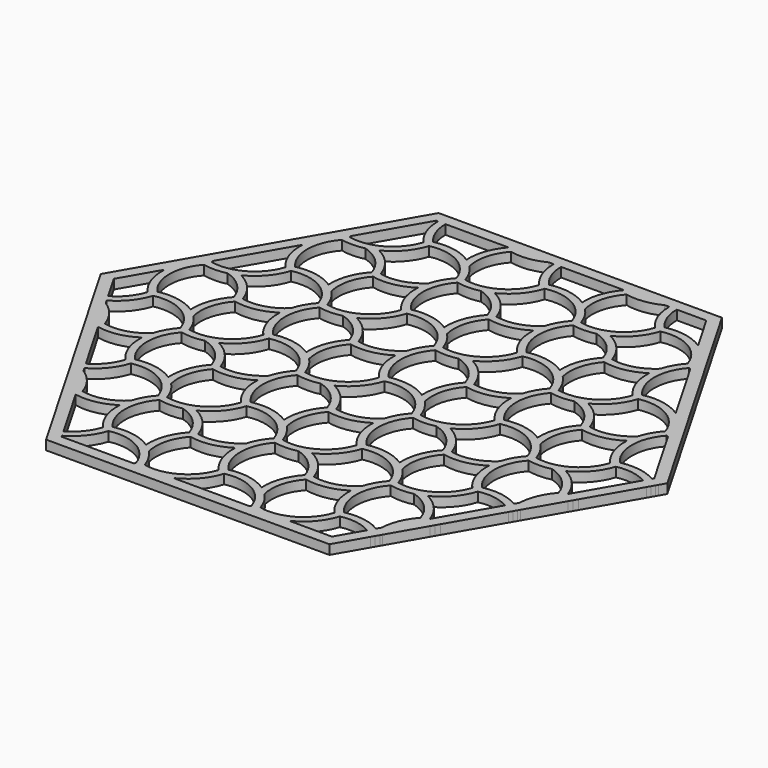
from build123d import *

# Parameters (mm, degrees)
F1_DEPTH = 2


with BuildPart() as f1:
    # F0 (on Top) → F1 (new body)
    with BuildSketch(Plane.XY):
        with BuildLine():
            ThreePointArc((-24.4948974278, 28.2842712475), (-16.9067069768, 29.2832754725), (-12.2474487139, 35.3553390593))
            ThreePointArc((-12.2474487139, 35.3553390593), (-15.1763809021, 42.4264068712), (-12.2474487139, 49.4974746831))
            ThreePointArc((-12.2474487139, 49.4974746831), (-16.9067069768, 55.5695382699), (-24.4948974278, 56.5685424949))
            ThreePointArc((-24.4948974278, 56.5685424949), (-29.1541556907, 50.4964789081), (-36.7423461417, 49.4974746831))
            ThreePointArc((-36.7423461417, 49.4974746831), (-39.6712783299, 42.4264068712), (-36.7423461417, 35.3553390593))
            ThreePointArc((-36.7423461417, 35.3553390593), (-29.1541556907, 34.3563348343), (-24.4948974278, 28.2842712475))
        make_face()
        with BuildLine():
            ThreePointArc((-36.4826087826, 36.242089814), (-38.8712783299, 42.4264068712), (-36.4826087826, 48.6107239284))
            ThreePointArc((-36.4826087826, 48.6107239284), (-34.0253641222, 48.3575009023), (-31.5748573601, 48.6692537387))
            ThreePointArc((-31.5748573601, 48.6692537387), (-30.9326704446, 48.8483852215), (-30.3027599763, 49.066799792))
            ThreePointArc((-30.3027599763, 49.066799792), (-29.8076116729, 49.2699966239), (-29.3231382191, 49.4974746831))
            ThreePointArc((-29.3231382191, 49.4974746831), (-25.9404111601, 52.1442868117), (-23.856817427, 55.9002279663))
            ThreePointArc((-23.856817427, 55.9002279663), (-17.3067069768, 54.8767179468), (-13.1452660739, 49.7159109091))
            ThreePointArc((-13.1452660739, 49.7159109091), (-14.5931859774, 47.7144861229), (-15.5484534825, 45.4364085966))
            ThreePointArc((-15.5484534825, 45.4364085966), (-15.7144145256, 44.7906926723), (-15.8402171931, 44.1359669195))
            ThreePointArc((-15.8402171931, 44.1359669195), (-15.9118177263, 43.6055574941), (-15.9570526752, 43.0722521461))
            ThreePointArc((-15.9570526752, 43.0722521461), (-15.3562096623, 38.8193185146), (-13.1452660739, 35.1369028333))
            ThreePointArc((-13.1452660739, 35.1369028333), (-17.3067069768, 29.9760957955), (-23.856817427, 28.9525857761))
            ThreePointArc((-23.856817427, 28.9525857761), (-24.8661421838, 31.2072335884), (-26.3613814409, 33.1735582783))
            ThreePointArc((-26.3613814409, 33.1735582783), (-26.8376073134, 33.6401427198), (-27.3417151141, 34.0764539021))
            ThreePointArc((-27.3417151141, 34.0764539021), (-27.7652628842, 34.4036664955), (-28.2045013891, 34.7094937844))
            ThreePointArc((-28.2045013891, 34.7094937844), (-32.1880714612, 36.3156152873), (-36.4826087826, 36.242089814))
        make_face(mode=Mode.SUBTRACT)
        with BuildLine():
            ThreePointArc((-24.4948974278, 56.5685424949), (-16.9067069768, 55.5695382699), (-12.2474487139, 49.4974746831))
            ThreePointArc((-12.2474487139, 49.4974746831), (-4.6592582629, 50.4964789081), (0, 56.5685424949))
            ThreePointArc((0, 56.5685424949), (-2.9289321881, 63.6396103068), (0, 70.7106781187))
            ThreePointArc((0, 70.7106781187), (-4.6592582629, 76.7827417055), (-12.2474487139, 77.7817459305))
            ThreePointArc((-12.2474487139, 77.7817459305), (-16.9067069768, 71.7096823437), (-24.4948974278, 70.7106781187))
            ThreePointArc((-24.4948974278, 70.7106781187), (-27.423829616, 63.6396103068), (-24.4948974278, 56.5685424949))
        make_face()
        with BuildLine():
            ThreePointArc((-0.89781736, 70.9291143447), (-2.3457372635, 68.9276895585), (-3.3010047685, 66.6496120322))
            ThreePointArc((-3.3010047685, 66.6496120322), (-3.4669658117, 66.0038961079), (-3.5927684791, 65.3491703551))
            ThreePointArc((-3.5927684791, 65.3491703551), (-3.6643690124, 64.8187609297), (-3.7096039613, 64.2854555817))
            ThreePointArc((-3.7096039613, 64.2854555817), (-3.1087609484, 60.0325219502), (-0.89781736, 56.3501062689))
            ThreePointArc((-0.89781736, 56.3501062689), (-5.0592582629, 51.1892992311), (-11.6093687131, 50.1657892117))
            ThreePointArc((-11.6093687131, 50.1657892117), (-12.6186934699, 52.420437024), (-14.113932727, 54.3867617139))
            ThreePointArc((-14.113932727, 54.3867617139), (-14.5901585994, 54.8533461554), (-15.0942664002, 55.2896573377))
            ThreePointArc((-15.0942664002, 55.2896573377), (-15.5178141703, 55.6168699311), (-15.9570526752, 55.92269722))
            ThreePointArc((-15.9570526752, 55.92269722), (-19.9406227472, 57.5288187229), (-24.2351600687, 57.4552932496))
            ThreePointArc((-24.2351600687, 57.4552932496), (-26.623829616, 63.6396103068), (-24.2351600687, 69.823927364))
            ThreePointArc((-24.2351600687, 69.823927364), (-21.7779154083, 69.5707043379), (-19.3274086462, 69.8824571743))
            ThreePointArc((-19.3274086462, 69.8824571743), (-18.6852217306, 70.0615886571), (-18.0553112624, 70.2800032276))
            ThreePointArc((-18.0553112624, 70.2800032276), (-17.560162959, 70.4832000595), (-17.0756895052, 70.7106781187))
            ThreePointArc((-17.0756895052, 70.7106781187), (-13.6929624462, 73.3574902473), (-11.6093687131, 77.1134314019))
            ThreePointArc((-11.6093687131, 77.1134314019), (-5.0592582629, 76.0899213824), (-0.89781736, 70.9291143447))
        make_face(mode=Mode.SUBTRACT)
        with BuildLine():
            ThreePointArc((0, 56.5685424949), (7.588190451, 55.5695382699), (12.2474487139, 49.4974746831))
            ThreePointArc((12.2474487139, 49.4974746831), (19.8356391649, 50.4964789081), (24.4948974278, 56.5685424949))
            ThreePointArc((24.4948974278, 56.5685424949), (21.5659652397, 63.6396103068), (24.4948974278, 70.7106781187))
            ThreePointArc((24.4948974278, 70.7106781187), (19.8356391649, 76.7827417055), (12.2474487139, 77.7817459305))
            ThreePointArc((12.2474487139, 77.7817459305), (7.588190451, 71.7096823437), (0, 70.7106781187))
            ThreePointArc((0, 70.7106781187), (-2.9289321881, 63.6396103068), (0, 56.5685424949))
        make_face()
        with BuildLine():
            ThreePointArc((12.8855287147, 50.1657892117), (11.8762039579, 52.420437024), (10.3809647008, 54.3867617139))
            ThreePointArc((10.3809647008, 54.3867617139), (9.9047388284, 54.8533461554), (9.4006310276, 55.2896573377))
            ThreePointArc((9.4006310276, 55.2896573377), (8.9770832575, 55.6168699311), (8.5378447526, 55.92269722))
            ThreePointArc((8.5378447526, 55.92269722), (4.5542746806, 57.5288187229), (0.2597373591, 57.4552932496))
            ThreePointArc((0.2597373591, 57.4552932496), (-2.1289321881, 63.6396103068), (0.2597373591, 69.823927364))
            ThreePointArc((0.2597373591, 69.823927364), (2.7169820195, 69.5707043379), (5.1674887816, 69.8824571743))
            ThreePointArc((5.1674887816, 69.8824571743), (5.8096756972, 70.0615886571), (6.4395861654, 70.2800032276))
            ThreePointArc((6.4395861654, 70.2800032276), (6.9347344688, 70.4832000595), (7.4192079226, 70.7106781187))
            ThreePointArc((7.4192079226, 70.7106781187), (10.8019349817, 73.3574902473), (12.8855287147, 77.1134314019))
            ThreePointArc((12.8855287147, 77.1134314019), (19.4356391649, 76.0899213824), (23.5970800679, 70.9291143447))
            ThreePointArc((23.5970800679, 70.9291143447), (22.1491601643, 68.9276895585), (21.1938926593, 66.6496120322))
            ThreePointArc((21.1938926593, 66.6496120322), (21.0279316162, 66.0038961079), (20.9021289487, 65.3491703551))
            ThreePointArc((20.9021289487, 65.3491703551), (20.8305284154, 64.8187609297), (20.7852934665, 64.2854555817))
            ThreePointArc((20.7852934665, 64.2854555817), (21.3861364795, 60.0325219502), (23.5970800679, 56.3501062689))
            ThreePointArc((23.5970800679, 56.3501062689), (19.4356391649, 51.1892992311), (12.8855287147, 50.1657892117))
        make_face(mode=Mode.SUBTRACT)
        with BuildLine():
            ThreePointArc((-12.2474487139, 35.3553390593), (-4.6592582629, 34.3563348343), (0, 28.2842712475))
            ThreePointArc((0, 28.2842712475), (7.588190451, 29.2832754725), (12.2474487139, 35.3553390593))
            ThreePointArc((12.2474487139, 35.3553390593), (9.3185165258, 42.4264068712), (12.2474487139, 49.4974746831))
            ThreePointArc((12.2474487139, 49.4974746831), (7.588190451, 55.5695382699), (0, 56.5685424949))
            ThreePointArc((0, 56.5685424949), (-4.6592582629, 50.4964789081), (-12.2474487139, 49.4974746831))
            ThreePointArc((-12.2474487139, 49.4974746831), (-15.1763809021, 42.4264068712), (-12.2474487139, 35.3553390593))
        make_face()
        with BuildLine():
            ThreePointArc((11.349631354, 49.7159109091), (9.9017114504, 47.7144861229), (8.9464439454, 45.4364085966))
            ThreePointArc((8.9464439454, 45.4364085966), (8.7804829023, 44.7906926723), (8.6546802348, 44.1359669195))
            ThreePointArc((8.6546802348, 44.1359669195), (8.5830797015, 43.6055574941), (8.5378447526, 43.0722521461))
            ThreePointArc((8.5378447526, 43.0722521461), (9.1386877656, 38.8193185146), (11.349631354, 35.1369028333))
            ThreePointArc((11.349631354, 35.1369028333), (7.188190451, 29.9760957955), (0.6380800008, 28.9525857761))
            ThreePointArc((0.6380800008, 28.9525857761), (-0.371244756, 31.2072335884), (-1.8664840131, 33.1735582783))
            ThreePointArc((-1.8664840131, 33.1735582783), (-2.3427098855, 33.6401427198), (-2.8468176863, 34.0764539021))
            ThreePointArc((-2.8468176863, 34.0764539021), (-3.2703654564, 34.4036664955), (-3.7096039613, 34.7094937844))
            ThreePointArc((-3.7096039613, 34.7094937844), (-7.6931740333, 36.3156152873), (-11.9877113548, 36.242089814))
            ThreePointArc((-11.9877113548, 36.242089814), (-14.3763809021, 42.4264068712), (-11.9877113548, 48.6107239284))
            ThreePointArc((-11.9877113548, 48.6107239284), (-9.5304666944, 48.3575009023), (-7.0799599323, 48.6692537387))
            ThreePointArc((-7.0799599323, 48.6692537387), (-6.4377730167, 48.8483852215), (-5.8078625485, 49.066799792))
            ThreePointArc((-5.8078625485, 49.066799792), (-5.3127142451, 49.2699966239), (-4.8282407913, 49.4974746831))
            ThreePointArc((-4.8282407913, 49.4974746831), (-1.4455137322, 52.1442868117), (0.6380800008, 55.9002279663))
            ThreePointArc((0.6380800008, 55.9002279663), (7.188190451, 54.8767179468), (11.349631354, 49.7159109091))
        make_face(mode=Mode.SUBTRACT)
        with BuildLine():
            ThreePointArc((12.2474487139, 49.4974746831), (9.3185165258, 42.4264068712), (12.2474487139, 35.3553390593))
            ThreePointArc((12.2474487139, 35.3553390593), (19.8356391649, 34.3563348343), (24.4948974278, 28.2842712475))
            ThreePointArc((24.4948974278, 28.2842712475), (32.0830878789, 29.2832754725), (36.7423461417, 35.3553390593))
            ThreePointArc((36.7423461417, 35.3553390593), (33.8134139536, 42.4264068712), (36.7423461417, 49.4974746831))
            ThreePointArc((36.7423461417, 49.4974746831), (32.0830878789, 55.5695382699), (24.4948974278, 56.5685424949))
            ThreePointArc((24.4948974278, 56.5685424949), (19.8356391649, 50.4964789081), (12.2474487139, 49.4974746831))
        make_face()
        with BuildLine():
            ThreePointArc((25.1329774287, 28.9525857761), (24.1236526718, 31.2072335884), (22.6284134148, 33.1735582783))
            ThreePointArc((22.6284134148, 33.1735582783), (22.1521875423, 33.6401427198), (21.6480797415, 34.0764539021))
            ThreePointArc((21.6480797415, 34.0764539021), (21.2245319714, 34.4036664955), (20.7852934665, 34.7094937844))
            ThreePointArc((20.7852934665, 34.7094937844), (16.8017233945, 36.3156152873), (12.507186073, 36.242089814))
            ThreePointArc((12.507186073, 36.242089814), (10.1185165258, 42.4264068712), (12.507186073, 48.6107239284))
            ThreePointArc((12.507186073, 48.6107239284), (14.9644307334, 48.3575009023), (17.4149374955, 48.6692537387))
            ThreePointArc((17.4149374955, 48.6692537387), (18.0571244111, 48.8483852215), (18.6870348794, 49.066799792))
            ThreePointArc((18.6870348794, 49.066799792), (19.1821831827, 49.2699966239), (19.6666566365, 49.4974746831))
            ThreePointArc((19.6666566365, 49.4974746831), (23.0493836956, 52.1442868117), (25.1329774287, 55.9002279663))
            ThreePointArc((25.1329774287, 55.9002279663), (31.6830878789, 54.8767179468), (35.8445287818, 49.7159109091))
            ThreePointArc((35.8445287818, 49.7159109091), (34.3966088782, 47.7144861229), (33.4413413732, 45.4364085966))
            ThreePointArc((33.4413413732, 45.4364085966), (33.2753803301, 44.7906926723), (33.1495776626, 44.1359669195))
            ThreePointArc((33.1495776626, 44.1359669195), (33.0779771293, 43.6055574941), (33.0327421804, 43.0722521461))
            ThreePointArc((33.0327421804, 43.0722521461), (33.6335851934, 38.8193185146), (35.8445287818, 35.1369028333))
            ThreePointArc((35.8445287818, 35.1369028333), (31.6830878789, 29.9760957955), (25.1329774287, 28.9525857761))
        make_face(mode=Mode.SUBTRACT)
        with BuildLine():
            ThreePointArc((-12.2474487139, 77.7817459305), (-4.6592582629, 76.7827417055), (0, 70.7106781187))
            ThreePointArc((0, 70.7106781187), (7.588190451, 71.7096823437), (12.2474487139, 77.7817459305))
            ThreePointArc((12.2474487139, 77.7817459305), (9.3185165258, 84.8528137424), (12.2474487139, 91.9238815543))
            ThreePointArc((12.2474487139, 91.9238815543), (7.588190451, 97.9959451411), (0, 98.9949493661))
            ThreePointArc((0, 98.9949493661), (-4.6592582629, 92.9228857793), (-12.2474487139, 91.9238815543))
            ThreePointArc((-12.2474487139, 91.9238815543), (-15.1763809021, 84.8528137424), (-12.2474487139, 77.7817459305))
        make_face()
        with BuildLine():
            ThreePointArc((0.6380800008, 71.3789926473), (-0.371244756, 73.6336404596), (-1.8664840131, 75.5999651495))
            ThreePointArc((-1.8664840131, 75.5999651495), (-2.3427098855, 76.066549591), (-2.8468176863, 76.5028607733))
            ThreePointArc((-2.8468176863, 76.5028607733), (-3.2703654564, 76.8300733667), (-3.7096039613, 77.1359006556))
            ThreePointArc((-3.7096039613, 77.1359006556), (-7.6931740333, 78.7420221585), (-11.9877113548, 78.6684966852))
            ThreePointArc((-11.9877113548, 78.6684966852), (-14.3763809021, 84.8528137424), (-11.9877113548, 91.0371307996))
            ThreePointArc((-11.9877113548, 91.0371307996), (-9.5304666944, 90.7839077735), (-7.0799599323, 91.0956606099))
            ThreePointArc((-7.0799599323, 91.0956606099), (-6.4377730167, 91.2747920927), (-5.8078625485, 91.4932066632))
            ThreePointArc((-5.8078625485, 91.4932066632), (-5.3127142451, 91.6964034951), (-4.8282407913, 91.9238815543))
            ThreePointArc((-4.8282407913, 91.9238815543), (-1.4455137322, 94.5706936829), (0.6380800008, 98.3266348375))
            ThreePointArc((0.6380800008, 98.3266348375), (7.188190451, 97.303124818), (11.349631354, 92.1423177803))
            ThreePointArc((11.349631354, 92.1423177803), (9.9017114504, 90.1408929941), (8.9464439454, 87.8628154678))
            ThreePointArc((8.9464439454, 87.8628154678), (8.7804829023, 87.2170995435), (8.6546802348, 86.5623737906))
            ThreePointArc((8.6546802348, 86.5623737906), (8.5830797015, 86.0319643653), (8.5378447526, 85.4986590173))
            ThreePointArc((8.5378447526, 85.4986590173), (9.1386877656, 81.2457253858), (11.349631354, 77.5633097045))
            ThreePointArc((11.349631354, 77.5633097045), (7.188190451, 72.4025026667), (0.6380800008, 71.3789926473))
        make_face(mode=Mode.SUBTRACT)
        with BuildLine():
            Line((-11.9953312015, 7.0070157729), (-7.3231853243, 7.0070157729))
            ThreePointArc((-7.3231853243, 7.0070157729), (-2.6807572434, 9.5678876966), (0, 14.1421356237))
            ThreePointArc((0, 14.1421356237), (-2.9289321881, 21.2132034356), (0, 28.2842712475))
            ThreePointArc((0, 28.2842712475), (-4.6592582629, 34.3563348343), (-12.2474487139, 35.3553390593))
            ThreePointArc((-12.2474487139, 35.3553390593), (-16.9067069768, 29.2832754725), (-24.4948974278, 28.2842712475))
            ThreePointArc((-24.4948974278, 28.2842712475), (-27.423829616, 21.2132034356), (-24.4948974278, 14.1421356237))
            ThreePointArc((-24.4948974278, 14.1421356237), (-16.9067069768, 13.1431313987), (-12.2474487139, 7.0710678119))
            ThreePointArc((-12.2474487139, 7.0710678119), (-12.1215982371, 7.0382219765), (-11.9953312015, 7.0070157729))
        make_face()
        with BuildLine():
            ThreePointArc((-24.2351600687, 15.0288863784), (-26.623829616, 21.2132034356), (-24.2351600687, 27.3975204928))
            ThreePointArc((-24.2351600687, 27.3975204928), (-21.7779154083, 27.1442974667), (-19.3274086462, 27.4560503031))
            ThreePointArc((-19.3274086462, 27.4560503031), (-18.6852217306, 27.6351817859), (-18.0553112624, 27.8535963564))
            ThreePointArc((-18.0553112624, 27.8535963564), (-17.560162959, 28.0567931883), (-17.0756895052, 28.2842712475))
            ThreePointArc((-17.0756895052, 28.2842712475), (-13.6929624462, 30.9310833761), (-11.6093687131, 34.6870245307))
            ThreePointArc((-11.6093687131, 34.6870245307), (-5.0592582629, 33.6635145113), (-0.89781736, 28.5027074735))
            ThreePointArc((-0.89781736, 28.5027074735), (-2.3457372635, 26.5012826873), (-3.3010047685, 24.223205161))
            ThreePointArc((-3.3010047685, 24.223205161), (-3.4669658117, 23.5774892367), (-3.5927684791, 22.9227634839))
            ThreePointArc((-3.5927684791, 22.9227634839), (-3.6643690124, 22.3923540585), (-3.7096039613, 21.8590487105))
            ThreePointArc((-3.7096039613, 21.8590487105), (-3.1087609484, 17.606115079), (-0.89781736, 13.9236993977))
            ThreePointArc((-0.89781736, 13.9236993977), (-5.0592582629, 8.7628923599), (-11.6093687131, 7.7393823405))
            ThreePointArc((-11.6093687131, 7.7393823405), (-12.6186934699, 9.9940301528), (-14.113932727, 11.9603548427))
            ThreePointArc((-14.113932727, 11.9603548427), (-14.5901585994, 12.4269392842), (-15.0942664002, 12.8632504665))
            ThreePointArc((-15.0942664002, 12.8632504665), (-15.5178141703, 13.1904630599), (-15.9570526752, 13.4962903488))
            ThreePointArc((-15.9570526752, 13.4962903488), (-19.9406227472, 15.1024118517), (-24.2351600687, 15.0288863784))
        make_face(mode=Mode.SUBTRACT)
        with BuildLine():
            ThreePointArc((0, 28.2842712475), (-2.9289321881, 21.2132034356), (0, 14.1421356237))
            ThreePointArc((0, 14.1421356237), (7.588190451, 13.1431313987), (12.2474487139, 7.0710678119))
            ThreePointArc((12.2474487139, 7.0710678119), (12.3732991907, 7.0382219765), (12.4995662263, 7.0070157729))
            Line((12.4995662263, 7.0070157729), (17.1717121035, 7.0070157729))
            ThreePointArc((17.1717121035, 7.0070157729), (21.8141401845, 9.5678876966), (24.4948974278, 14.1421356237))
            ThreePointArc((24.4948974278, 14.1421356237), (21.5659652397, 21.2132034356), (24.4948974278, 28.2842712475))
            ThreePointArc((24.4948974278, 28.2842712475), (19.8356391649, 34.3563348343), (12.2474487139, 35.3553390593))
            ThreePointArc((12.2474487139, 35.3553390593), (7.588190451, 29.2832754725), (0, 28.2842712475))
        make_face()
        with BuildLine():
            ThreePointArc((23.5970800679, 28.5027074735), (22.1491601643, 26.5012826873), (21.1938926593, 24.223205161))
            ThreePointArc((21.1938926593, 24.223205161), (21.0279316162, 23.5774892367), (20.9021289487, 22.9227634839))
            ThreePointArc((20.9021289487, 22.9227634839), (20.8305284154, 22.3923540585), (20.7852934665, 21.8590487105))
            ThreePointArc((20.7852934665, 21.8590487105), (21.3861364795, 17.606115079), (23.5970800679, 13.9236993977))
            ThreePointArc((23.5970800679, 13.9236993977), (19.4356391649, 8.7628923599), (12.8855287147, 7.7393823405))
            ThreePointArc((12.8855287147, 7.7393823405), (11.8762039579, 9.9940301528), (10.3809647008, 11.9603548427))
            ThreePointArc((10.3809647008, 11.9603548427), (9.9047388284, 12.4269392842), (9.4006310276, 12.8632504665))
            ThreePointArc((9.4006310276, 12.8632504665), (8.9770832575, 13.1904630599), (8.5378447526, 13.4962903488))
            ThreePointArc((8.5378447526, 13.4962903488), (4.5542746806, 15.1024118517), (0.2597373591, 15.0288863784))
            ThreePointArc((0.2597373591, 15.0288863784), (-2.1289321881, 21.2132034356), (0.2597373591, 27.3975204928))
            ThreePointArc((0.2597373591, 27.3975204928), (2.7169820195, 27.1442974667), (5.1674887816, 27.4560503031))
            ThreePointArc((5.1674887816, 27.4560503031), (5.8096756972, 27.6351817859), (6.4395861654, 27.8535963564))
            ThreePointArc((6.4395861654, 27.8535963564), (6.9347344688, 28.0567931883), (7.4192079226, 28.2842712475))
            ThreePointArc((7.4192079226, 28.2842712475), (10.8019349817, 30.9310833761), (12.8855287147, 34.6870245307))
            ThreePointArc((12.8855287147, 34.6870245307), (19.4356391649, 33.6635145113), (23.5970800679, 28.5027074735))
        make_face(mode=Mode.SUBTRACT)
        with BuildLine():
            ThreePointArc((24.4948974278, 70.7106781187), (21.5659652397, 63.6396103068), (24.4948974278, 56.5685424949))
            ThreePointArc((24.4948974278, 56.5685424949), (32.0830878789, 55.5695382699), (36.7423461417, 49.4974746831))
            ThreePointArc((36.7423461417, 49.4974746831), (44.3305365928, 50.4964789081), (48.9897948557, 56.5685424949))
            ThreePointArc((48.9897948557, 56.5685424949), (46.0608626675, 63.6396103068), (48.9897948557, 70.7106781187))
            ThreePointArc((48.9897948557, 70.7106781187), (48.9553171187, 70.8360830369), (48.9192113397, 70.9610289476))
            Line((48.9192113397, 70.9610289476), (46.5831228244, 75.0072529471))
            ThreePointArc((46.5831228244, 75.0072529471), (42.0441319621, 77.7472681935), (36.7423461417, 77.7817459305))
            ThreePointArc((36.7423461417, 77.7817459305), (32.0830878789, 71.7096823437), (24.4948974278, 70.7106781187))
        make_face()
        with BuildLine():
            ThreePointArc((48.0919774957, 70.9291143447), (46.6440575921, 68.9276895585), (45.6887900871, 66.6496120322))
            ThreePointArc((45.6887900871, 66.6496120322), (45.522829044, 66.0038961079), (45.3970263765, 65.3491703551))
            ThreePointArc((45.3970263765, 65.3491703551), (45.3254258432, 64.8187609297), (45.2801908944, 64.2854555817))
            ThreePointArc((45.2801908944, 64.2854555817), (45.8810339073, 60.0325219502), (48.0919774957, 56.3501062689))
            ThreePointArc((48.0919774957, 56.3501062689), (43.9305365928, 51.1892992311), (37.3804261426, 50.1657892117))
            ThreePointArc((37.3804261426, 50.1657892117), (36.3711013857, 52.420437024), (34.8758621287, 54.3867617139))
            ThreePointArc((34.8758621287, 54.3867617139), (34.3996362562, 54.8533461554), (33.8955284555, 55.2896573377))
            ThreePointArc((33.8955284555, 55.2896573377), (33.4719806854, 55.6168699311), (33.0327421804, 55.92269722))
            ThreePointArc((33.0327421804, 55.92269722), (29.0491721084, 57.5288187229), (24.754634787, 57.4552932496))
            ThreePointArc((24.754634787, 57.4552932496), (22.3659652397, 63.6396103068), (24.754634787, 69.823927364))
            ThreePointArc((24.754634787, 69.823927364), (27.2118794474, 69.5707043379), (29.6623862094, 69.8824571743))
            ThreePointArc((29.6623862094, 69.8824571743), (30.304573125, 70.0615886571), (30.9344835933, 70.2800032276))
            ThreePointArc((30.9344835933, 70.2800032276), (31.4296318966, 70.4832000595), (31.9141053504, 70.7106781187))
            ThreePointArc((31.9141053504, 70.7106781187), (35.2968324095, 73.3574902473), (37.3804261426, 77.1134314019))
            ThreePointArc((37.3804261426, 77.1134314019), (43.9305365928, 76.0899213824), (48.0919774957, 70.9291143447))
        make_face(mode=Mode.SUBTRACT)
        with BuildLine():
            ThreePointArc((12.2474487139, 77.7817459305), (19.8356391649, 76.7827417055), (24.4948974278, 70.7106781187))
            ThreePointArc((24.4948974278, 70.7106781187), (32.0830878789, 71.7096823437), (36.7423461417, 77.7817459305))
            ThreePointArc((36.7423461417, 77.7817459305), (33.8134139536, 84.8528137424), (36.7423461417, 91.9238815543))
            ThreePointArc((36.7423461417, 91.9238815543), (36.7078684048, 92.0492864725), (36.6717626258, 92.1742323832))
            Line((36.6717626258, 92.1742323832), (34.3356741105, 96.2204563827))
            ThreePointArc((34.3356741105, 96.2204563827), (29.7966832482, 98.9604716291), (24.4948974278, 98.9949493661))
            ThreePointArc((24.4948974278, 98.9949493661), (19.8356391649, 92.9228857793), (12.2474487139, 91.9238815543))
            ThreePointArc((12.2474487139, 91.9238815543), (9.3185165258, 84.8528137424), (12.2474487139, 77.7817459305))
        make_face()
        with BuildLine():
            ThreePointArc((35.8445287818, 92.1423177803), (34.3966088782, 90.1408929941), (33.4413413732, 87.8628154678))
            ThreePointArc((33.4413413732, 87.8628154678), (33.2753803301, 87.2170995435), (33.1495776626, 86.5623737906))
            ThreePointArc((33.1495776626, 86.5623737906), (33.0779771293, 86.0319643653), (33.0327421804, 85.4986590173))
            ThreePointArc((33.0327421804, 85.4986590173), (33.6335851934, 81.2457253858), (35.8445287818, 77.5633097045))
            ThreePointArc((35.8445287818, 77.5633097045), (31.6830878789, 72.4025026667), (25.1329774287, 71.3789926473))
            ThreePointArc((25.1329774287, 71.3789926473), (24.1236526718, 73.6336404596), (22.6284134148, 75.5999651495))
            ThreePointArc((22.6284134148, 75.5999651495), (22.1521875423, 76.066549591), (21.6480797415, 76.5028607733))
            ThreePointArc((21.6480797415, 76.5028607733), (21.2245319714, 76.8300733667), (20.7852934665, 77.1359006556))
            ThreePointArc((20.7852934665, 77.1359006556), (16.8017233945, 78.7420221585), (12.507186073, 78.6684966852))
            ThreePointArc((12.507186073, 78.6684966852), (10.1185165258, 84.8528137424), (12.507186073, 91.0371307996))
            ThreePointArc((12.507186073, 91.0371307996), (14.9644307334, 90.7839077735), (17.4149374955, 91.0956606099))
            ThreePointArc((17.4149374955, 91.0956606099), (18.0571244111, 91.2747920927), (18.6870348794, 91.4932066632))
            ThreePointArc((18.6870348794, 91.4932066632), (19.1821831827, 91.6964034951), (19.6666566365, 91.9238815543))
            ThreePointArc((19.6666566365, 91.9238815543), (23.0493836956, 94.5706936829), (25.1329774287, 98.3266348375))
            ThreePointArc((25.1329774287, 98.3266348375), (31.6830878789, 97.303124818), (35.8445287818, 92.1423177803))
        make_face(mode=Mode.SUBTRACT)
        with BuildLine():
            ThreePointArc((-36.7423461417, 77.7817459305), (-29.1541556907, 76.7827417055), (-24.4948974278, 70.7106781187))
            ThreePointArc((-24.4948974278, 70.7106781187), (-16.9067069768, 71.7096823437), (-12.2474487139, 77.7817459305))
            ThreePointArc((-12.2474487139, 77.7817459305), (-15.1763809021, 84.8528137424), (-12.2474487139, 91.9238815543))
            ThreePointArc((-12.2474487139, 91.9238815543), (-16.9067069768, 97.9959451411), (-24.4948974278, 98.9949493661))
            ThreePointArc((-24.4948974278, 98.9949493661), (-29.1541556907, 92.9228857793), (-36.7423461417, 91.9238815543))
            ThreePointArc((-36.7423461417, 91.9238815543), (-36.8337111182, 91.831320499), (-36.9238645615, 91.7375790218))
            Line((-36.9238645615, 91.7375790218), (-39.2599530768, 87.6913550224))
            ThreePointArc((-39.2599530768, 87.6913550224), (-39.3633804558, 82.3904660048), (-36.7423461417, 77.7817459305))
        make_face()
        with BuildLine():
            ThreePointArc((-13.1452660739, 92.1423177803), (-14.5931859774, 90.1408929941), (-15.5484534825, 87.8628154678))
            ThreePointArc((-15.5484534825, 87.8628154678), (-15.7144145256, 87.2170995435), (-15.8402171931, 86.5623737906))
            ThreePointArc((-15.8402171931, 86.5623737906), (-15.9118177263, 86.0319643653), (-15.9570526752, 85.4986590173))
            ThreePointArc((-15.9570526752, 85.4986590173), (-15.3562096623, 81.2457253858), (-13.1452660739, 77.5633097045))
            ThreePointArc((-13.1452660739, 77.5633097045), (-17.3067069768, 72.4025026667), (-23.856817427, 71.3789926473))
            ThreePointArc((-23.856817427, 71.3789926473), (-24.8661421838, 73.6336404596), (-26.3613814409, 75.5999651495))
            ThreePointArc((-26.3613814409, 75.5999651495), (-26.8376073134, 76.066549591), (-27.3417151141, 76.5028607733))
            ThreePointArc((-27.3417151141, 76.5028607733), (-27.7652628842, 76.8300733667), (-28.2045013891, 77.1359006556))
            ThreePointArc((-28.2045013891, 77.1359006556), (-32.1880714612, 78.7420221585), (-36.4826087826, 78.6684966852))
            ThreePointArc((-36.4826087826, 78.6684966852), (-38.8712783299, 84.8528137424), (-36.4826087826, 91.0371307996))
            ThreePointArc((-36.4826087826, 91.0371307996), (-34.0253641222, 90.7839077735), (-31.5748573601, 91.0956606099))
            ThreePointArc((-31.5748573601, 91.0956606099), (-30.9326704446, 91.2747920927), (-30.3027599763, 91.4932066632))
            ThreePointArc((-30.3027599763, 91.4932066632), (-29.8076116729, 91.6964034951), (-29.3231382191, 91.9238815543))
            ThreePointArc((-29.3231382191, 91.9238815543), (-25.9404111601, 94.5706936829), (-23.856817427, 98.3266348375))
            ThreePointArc((-23.856817427, 98.3266348375), (-17.3067069768, 97.303124818), (-13.1452660739, 92.1423177803))
        make_face(mode=Mode.SUBTRACT)
        with BuildLine():
            ThreePointArc((-36.7423461417, 49.4974746831), (-29.1541556907, 50.4964789081), (-24.4948974278, 56.5685424949))
            ThreePointArc((-24.4948974278, 56.5685424949), (-27.423829616, 63.6396103068), (-24.4948974278, 70.7106781187))
            ThreePointArc((-24.4948974278, 70.7106781187), (-29.1541556907, 76.7827417055), (-36.7423461417, 77.7817459305))
            ThreePointArc((-36.7423461417, 77.7817459305), (-41.4016044046, 71.7096823437), (-48.9897948557, 70.7106781187))
            ThreePointArc((-48.9897948557, 70.7106781187), (-49.0811598322, 70.6181170634), (-49.1713132754, 70.5243755862))
            Line((-49.1713132754, 70.5243755862), (-51.5074017907, 66.4781515868))
            ThreePointArc((-51.5074017907, 66.4781515868), (-51.6108291697, 61.1772625692), (-48.9897948557, 56.5685424949))
            ThreePointArc((-48.9897948557, 56.5685424949), (-41.4016044046, 55.5695382699), (-36.7423461417, 49.4974746831))
        make_face()
        with BuildLine():
            ThreePointArc((-48.7300574965, 57.4552932496), (-51.1187270438, 63.6396103068), (-48.7300574965, 69.823927364))
            ThreePointArc((-48.7300574965, 69.823927364), (-46.2728128361, 69.5707043379), (-43.8223060741, 69.8824571743))
            ThreePointArc((-43.8223060741, 69.8824571743), (-43.1801191585, 70.0615886571), (-42.5502086902, 70.2800032276))
            ThreePointArc((-42.5502086902, 70.2800032276), (-42.0550603869, 70.4832000595), (-41.5705869331, 70.7106781187))
            ThreePointArc((-41.5705869331, 70.7106781187), (-38.187859874, 73.3574902473), (-36.1042661409, 77.1134314019))
            ThreePointArc((-36.1042661409, 77.1134314019), (-29.5541556907, 76.0899213824), (-25.3927147878, 70.9291143447))
            ThreePointArc((-25.3927147878, 70.9291143447), (-26.8406346914, 68.9276895585), (-27.7959021964, 66.6496120322))
            ThreePointArc((-27.7959021964, 66.6496120322), (-27.9618632395, 66.0038961079), (-28.087665907, 65.3491703551))
            ThreePointArc((-28.087665907, 65.3491703551), (-28.1592664403, 64.8187609297), (-28.2045013891, 64.2854555817))
            ThreePointArc((-28.2045013891, 64.2854555817), (-27.6036583762, 60.0325219502), (-25.3927147878, 56.3501062689))
            ThreePointArc((-25.3927147878, 56.3501062689), (-29.5541556907, 51.1892992311), (-36.1042661409, 50.1657892117))
            ThreePointArc((-36.1042661409, 50.1657892117), (-37.1135908978, 52.420437024), (-38.6088301548, 54.3867617139))
            ThreePointArc((-38.6088301548, 54.3867617139), (-39.0850560273, 54.8533461554), (-39.589163828, 55.2896573377))
            ThreePointArc((-39.589163828, 55.2896573377), (-40.0127115981, 55.6168699311), (-40.4519501031, 55.92269722))
            ThreePointArc((-40.4519501031, 55.92269722), (-44.4355201751, 57.5288187229), (-48.7300574965, 57.4552932496))
        make_face(mode=Mode.SUBTRACT)
        with BuildLine():
            ThreePointArc((-41.4571765808, 29.2514277222), (-38.4876076121, 31.8305388538), (-36.7423461417, 35.3553390593))
            ThreePointArc((-36.7423461417, 35.3553390593), (-39.6712783299, 42.4264068712), (-36.7423461417, 49.4974746831))
            ThreePointArc((-36.7423461417, 49.4974746831), (-41.4016044046, 55.5695382699), (-48.9897948557, 56.5685424949))
            ThreePointArc((-48.9897948557, 56.5685424949), (-50.735056326, 53.0437422894), (-53.7046252947, 50.4646311578))
            Line((-53.7046252947, 50.4646311578), (-53.3046176973, 49.7717976756))
            ThreePointArc((-53.3046176973, 49.7717976756), (-50.2493099404, 52.3681900581), (-48.3517148548, 55.9002279663))
            ThreePointArc((-48.3517148548, 55.9002279663), (-41.8016044046, 54.8767179468), (-37.6401635017, 49.7159109091))
            ThreePointArc((-37.6401635017, 49.7159109091), (-39.0880834053, 47.7144861229), (-40.0433509103, 45.4364085966))
            ThreePointArc((-40.0433509103, 45.4364085966), (-40.2093119534, 44.7906926723), (-40.3351146209, 44.1359669195))
            ThreePointArc((-40.3351146209, 44.1359669195), (-40.4067151542, 43.6055574941), (-40.4519501031, 43.0722521461))
            ThreePointArc((-40.4519501031, 43.0722521461), (-39.8511070901, 38.8193185146), (-37.6401635017, 35.1369028333))
            ThreePointArc((-37.6401635017, 35.1369028333), (-39.2600112955, 32.1437322843), (-41.8571854996, 29.944263493))
            Line((-41.8571854996, 29.944263493), (-41.4571765808, 29.2514277222))
        make_face()
        with BuildLine():
            ThreePointArc((-29.2097278669, 8.0382242866), (-26.2401588982, 10.6173354182), (-24.4948974278, 14.1421356237))
            ThreePointArc((-24.4948974278, 14.1421356237), (-27.423829616, 21.2132034356), (-24.4948974278, 28.2842712475))
            ThreePointArc((-24.4948974278, 28.2842712475), (-29.1541556907, 34.3563348343), (-36.7423461417, 35.3553390593))
            ThreePointArc((-36.7423461417, 35.3553390593), (-38.4876076121, 31.8305388538), (-41.4571765808, 29.2514277222))
            Line((-41.4571765808, 29.2514277222), (-41.0571689834, 28.55859424))
            ThreePointArc((-41.0571689834, 28.55859424), (-38.0018612264, 31.1549866225), (-36.1042661409, 34.6870245307))
            ThreePointArc((-36.1042661409, 34.6870245307), (-29.5541556907, 33.6635145113), (-25.3927147878, 28.5027074735))
            ThreePointArc((-25.3927147878, 28.5027074735), (-26.8406346914, 26.5012826873), (-27.7959021964, 24.223205161))
            ThreePointArc((-27.7959021964, 24.223205161), (-27.9618632395, 23.5774892367), (-28.087665907, 22.9227634839))
            ThreePointArc((-28.087665907, 22.9227634839), (-28.1592664403, 22.3923540585), (-28.2045013891, 21.8590487105))
            ThreePointArc((-28.2045013891, 21.8590487105), (-27.6036583762, 17.606115079), (-25.3927147878, 13.9236993977))
            ThreePointArc((-25.3927147878, 13.9236993977), (-27.0125625816, 10.9305288487), (-29.6097367857, 8.7310600574))
            Line((-29.6097367857, 8.7310600574), (-29.2097278669, 8.0382242866))
        make_face()
        with BuildLine():
            ThreePointArc((36.7423461417, 49.4974746831), (33.8134139536, 42.4264068712), (36.7423461417, 35.3553390593))
            ThreePointArc((36.7423461417, 35.3553390593), (40.6675433982, 35.6062983925), (44.3859036417, 34.3241317931))
            Line((44.3859036417, 34.3241317931), (44.7859112391, 35.0169652753))
            ThreePointArc((44.7859112391, 35.0169652753), (41.0097155992, 36.364743218), (37.0020835009, 36.242089814))
            ThreePointArc((37.0020835009, 36.242089814), (34.6134139536, 42.4264068712), (37.0020835009, 48.6107239284))
            ThreePointArc((37.0020835009, 48.6107239284), (39.4593281613, 48.3575009023), (41.9098349234, 48.6692537387))
            ThreePointArc((41.9098349234, 48.6692537387), (42.5520218389, 48.8483852215), (43.1819323072, 49.066799792))
            ThreePointArc((43.1819323072, 49.066799792), (43.6770806106, 49.2699966239), (44.1615540644, 49.4974746831))
            ThreePointArc((44.1615540644, 49.4974746831), (47.5442811234, 52.1442868117), (49.6278748565, 55.9002279663))
            ThreePointArc((49.6278748565, 55.9002279663), (53.0299604867, 55.9939839011), (56.2333434368, 54.8444994579))
            Line((56.2333434368, 54.8444994579), (56.6333523556, 55.5373352287))
            ThreePointArc((56.6333523556, 55.5373352287), (52.9149921121, 56.8195018281), (48.9897948557, 56.5685424949))
            ThreePointArc((48.9897948557, 56.5685424949), (44.3305365928, 50.4964789081), (36.7423461417, 49.4974746831))
        make_face()
        with BuildLine():
            ThreePointArc((24.4948974278, 28.2842712475), (21.5659652397, 21.2132034356), (24.4948974278, 14.1421356237))
            ThreePointArc((24.4948974278, 14.1421356237), (28.4200946843, 14.393094957), (32.1384549278, 13.1109283575))
            Line((32.1384549278, 13.1109283575), (32.5384625252, 13.8037618397))
            ThreePointArc((32.5384625252, 13.8037618397), (28.7622668853, 15.1515397824), (24.754634787, 15.0288863784))
            ThreePointArc((24.754634787, 15.0288863784), (22.3659652397, 21.2132034356), (24.754634787, 27.3975204928))
            ThreePointArc((24.754634787, 27.3975204928), (27.2118794474, 27.1442974667), (29.6623862094, 27.4560503031))
            ThreePointArc((29.6623862094, 27.4560503031), (30.304573125, 27.6351817859), (30.9344835933, 27.8535963564))
            ThreePointArc((30.9344835933, 27.8535963564), (31.4296318966, 28.0567931883), (31.9141053504, 28.2842712475))
            ThreePointArc((31.9141053504, 28.2842712475), (35.2968324095, 30.9310833761), (37.3804261426, 34.6870245307))
            ThreePointArc((37.3804261426, 34.6870245307), (40.7825117727, 34.7807804655), (43.9858947229, 33.6312960223))
            Line((43.9858947229, 33.6312960223), (44.3859036417, 34.3241317931))
            ThreePointArc((44.3859036417, 34.3241317931), (40.6675433982, 35.6062983925), (36.7423461417, 35.3553390593))
            ThreePointArc((36.7423461417, 35.3553390593), (32.0830878789, 29.2832754725), (24.4948974278, 28.2842712475))
        make_face()
        with BuildLine():
            ThreePointArc((-24.4948974278, 98.9949493661), (-16.9067069768, 97.9959451411), (-12.2474487139, 91.9238815543))
            ThreePointArc((-12.2474487139, 91.9238815543), (-4.6592582629, 92.9228857793), (0, 98.9949493661))
            ThreePointArc((0, 98.9949493661), (-2.1799350756, 102.2687885074), (-2.9287270848, 106.1300642271))
            Line((-2.9287270848, 106.1300642271), (-3.7287422779, 106.1300642271))
            ThreePointArc((-3.7287422779, 106.1300642271), (-3.0078537005, 102.185895898), (-0.89781736, 98.7765131401))
            ThreePointArc((-0.89781736, 98.7765131401), (-5.0592582629, 93.6157061023), (-11.6093687131, 92.5921960829))
            ThreePointArc((-11.6093687131, 92.5921960829), (-12.6186934699, 94.8468438952), (-14.113932727, 96.8131685851))
            ThreePointArc((-14.113932727, 96.8131685851), (-14.5901585994, 97.2797530266), (-15.0942664002, 97.7160642089))
            ThreePointArc((-15.0942664002, 97.7160642089), (-15.5178141703, 98.0432768023), (-15.9570526752, 98.3491040912))
            ThreePointArc((-15.9570526752, 98.3491040912), (-19.9406227472, 99.9552255941), (-24.2351600687, 99.8817001208))
            ThreePointArc((-24.2351600687, 99.8817001208), (-26.017397237, 102.7811129871), (-26.6236066772, 106.1300642271))
            Line((-26.6236066772, 106.1300642271), (-27.4236245126, 106.1300642271))
            ThreePointArc((-27.4236245126, 106.1300642271), (-26.6748325034, 102.2687885074), (-24.4948974278, 98.9949493661))
        make_face()
        with BuildLine():
            ThreePointArc((0, 98.9949493661), (7.588190451, 97.9959451411), (12.2474487139, 91.9238815543))
            ThreePointArc((12.2474487139, 91.9238815543), (19.8356391649, 92.9228857793), (24.4948974278, 98.9949493661))
            ThreePointArc((24.4948974278, 98.9949493661), (22.3149623523, 102.2687885074), (21.566170343, 106.1300642271))
            Line((21.566170343, 106.1300642271), (20.7661551499, 106.1300642271))
            ThreePointArc((20.7661551499, 106.1300642271), (21.4870437273, 102.185895898), (23.5970800679, 98.7765131401))
            ThreePointArc((23.5970800679, 98.7765131401), (19.4356391649, 93.6157061023), (12.8855287147, 92.5921960829))
            ThreePointArc((12.8855287147, 92.5921960829), (11.8762039579, 94.8468438952), (10.3809647008, 96.8131685851))
            ThreePointArc((10.3809647008, 96.8131685851), (9.9047388284, 97.2797530266), (9.4006310276, 97.7160642089))
            ThreePointArc((9.4006310276, 97.7160642089), (8.9770832575, 98.0432768023), (8.5378447526, 98.3491040912))
            ThreePointArc((8.5378447526, 98.3491040912), (4.5542746806, 99.9552255941), (0.2597373591, 99.8817001208))
            ThreePointArc((0.2597373591, 99.8817001208), (-1.5224998091, 102.7811129871), (-2.1287092493, 106.1300642271))
            Line((-2.1287092493, 106.1300642271), (-2.9287270848, 106.1300642271))
            ThreePointArc((-2.9287270848, 106.1300642271), (-2.1799350756, 102.2687885074), (0, 98.9949493661))
        make_face()
        with BuildLine():
            ThreePointArc((-56.3510413016, 50.2483581397), (-55.1977730309, 50.6286226186), (-54.1046342135, 51.1574669286))
            Line((-54.1046342135, 51.1574669286), (-57.2287187079, 56.56854))
            Line((-57.2287187079, 56.56854), (-52.8178624101, 64.2083672127))
            ThreePointArc((-52.8178624101, 64.2083672127), (-54.5635939476, 63.3014177265), (-56.4448817479, 62.7261854396))
            Line((-56.4448817479, 62.7261854396), (-60, 56.56854))
            Line((-60, 56.56854), (-56.3510413016, 50.2483581397))
        make_face()
        with BuildLine():
            ThreePointArc((22.7020794022, 108.5300642271), (22.4547644775, 107.3411723336), (22.3661881785, 106.1300642271))
            Line((22.3661881785, 106.1300642271), (28.6143593539, 106.1300642271))
            Line((28.6143593539, 106.1300642271), (33.0252134911, 98.4902407568))
            ThreePointArc((33.0252134911, 98.4902407568), (33.1126379648, 100.4555633595), (33.5551160915, 102.3724225298))
            Line((33.5551160915, 102.3724225298), (30, 108.5300642271))
            Line((30, 108.5300642271), (22.7020794022, 108.5300642271))
        make_face()
        with BuildLine():
            ThreePointArc((19.7926561631, 7.0070157729), (21.4509611886, 5.9486423647), (22.8897689997, 4.6070157729))
            Line((22.8897689997, 4.6070157729), (30, 4.6070157729))
            Line((30, 4.6070157729), (33.6489608591, 10.9272013757))
            ThreePointArc((33.6489608591, 10.9272013757), (32.7430080248, 11.7358287561), (31.738446009, 12.4180925867))
            Line((31.738446009, 12.4180925867), (28.6143593539, 7.0070157729))
            Line((28.6143593539, 7.0070157729), (19.7926561631, 7.0070157729))
        make_face()
        with BuildLine():
            ThreePointArc((-37.5277688705, 95.4915860758), (-36.7915387792, 94.2638386937), (-36.2241603077, 92.9495023397))
            Line((-36.2241603077, 92.9495023397), (-28.6143593539, 106.1300642271))
            Line((-28.6143593539, 106.1300642271), (-28.2236397058, 106.1300642271))
            ThreePointArc((-28.2236397058, 106.1300642271), (-28.2179910773, 106.4210923062), (-28.2045013891, 106.7118624529))
            ThreePointArc((-28.2045013891, 106.7118624529), (-30.0033667154, 105.7547713973), (-31.94998432, 105.1525923108))
            Line((-31.94998432, 105.1525923108), (-37.5277688705, 95.4915860758))
        make_face()
        with BuildLine():
            Line((57.2287187079, 56.56854), (57.033359953, 56.2301687109))
            ThreePointArc((57.033359953, 56.2301687109), (57.2825717076, 56.0797637176), (57.5276396083, 55.92269722))
            ThreePointArc((57.5276396083, 55.92269722), (57.5982071035, 57.9591058183), (58.0500135193, 59.9460156586))
            Line((58.0500135193, 59.9460156586), (52.4722289688, 69.6070218937))
            ThreePointArc((52.4722289688, 69.6070218937), (51.0408535009, 69.5833016226), (49.6189155935, 69.7491056297))
            Line((49.6189155935, 69.7491056297), (57.2287187079, 56.56854))
        make_face()
        with BuildLine():
            Line((-26.100025856, 4.6070157729), (-14.9444618634, 4.6070157729))
            ThreePointArc((-14.9444618634, 4.6070157729), (-14.2493171779, 5.8584833647), (-13.3947584766, 7.0070157729))
            Line((-13.3947584766, 7.0070157729), (-28.6143593539, 7.0070157729))
            Line((-28.6143593539, 7.0070157729), (-28.8097202695, 7.3453908044))
            ThreePointArc((-28.8097202695, 7.3453908044), (-29.0645806918, 7.2047695907), (-29.3231382191, 7.0710678119))
            ThreePointArc((-29.3231382191, 7.0710678119), (-27.5948383948, 5.9917487452), (-26.100025856, 4.6070157729))
        make_face()
        with BuildLine():
            Line((37.3714668796, 90.9623090653), (45.272662205, 77.2770373212))
            ThreePointArc((45.272662205, 77.2770373212), (45.3600866787, 79.2423599239), (45.8025648054, 81.1592190942))
            Line((45.8025648054, 81.1592190942), (40.2247802549, 90.8202253293))
            ThreePointArc((40.2247802549, 90.8202253293), (38.793404787, 90.7965050582), (37.3714668796, 90.9623090653))
        make_face()
        with BuildLine():
            ThreePointArc((-49.7752175844, 74.2783826402), (-49.0389874931, 73.0506352581), (-48.4716090216, 71.7362989041))
            Line((-48.4716090216, 71.7362989041), (-40.5704136962, 85.4215706483))
            ThreePointArc((-40.5704136962, 85.4215706483), (-42.3161452336, 84.5146211621), (-44.1974330339, 83.9393888752))
            Line((-44.1974330339, 83.9393888752), (-49.7752175844, 74.2783826402))
        make_face()
        with BuildLine():
            ThreePointArc((-4.7022412648, 7.0070157729), (-3.0439362392, 5.9486423647), (-1.6051284282, 4.6070157729))
            Line((-1.6051284282, 4.6070157729), (9.5504355644, 4.6070157729))
            ThreePointArc((9.5504355644, 4.6070157729), (10.2455802499, 5.8584833647), (11.1001389512, 7.0070157729))
            Line((11.1001389512, 7.0070157729), (-4.7022412648, 7.0070157729))
        make_face()
        with BuildLine():
            ThreePointArc((-1.7928180256, 108.5300642271), (-2.0401329503, 107.3411723336), (-2.1287092493, 106.1300642271))
            Line((-2.1287092493, 106.1300642271), (11.2111041198, 106.1300642271))
            ThreePointArc((11.2111041198, 106.1300642271), (11.2799970752, 106.2075913954), (11.349631354, 106.284453404))
            ThreePointArc((11.349631354, 106.284453404), (10.8895052832, 107.4437026778), (10.2768116696, 108.5300642271))
            Line((10.2768116696, 108.5300642271), (-1.7928180256, 108.5300642271))
        make_face()
        with BuildLine():
            ThreePointArc((-26.2877154534, 108.5300642271), (-26.5350303782, 107.3411723336), (-26.6236066772, 106.1300642271))
            Line((-26.6236066772, 106.1300642271), (-13.2837933081, 106.1300642271))
            ThreePointArc((-13.2837933081, 106.1300642271), (-13.2149003526, 106.2075913954), (-13.1452660739, 106.284453404))
            ThreePointArc((-13.1452660739, 106.284453404), (-13.6053921447, 107.4437026778), (-14.2180857582, 108.5300642271))
            Line((-14.2180857582, 108.5300642271), (-26.2877154534, 108.5300642271))
        make_face()
        with BuildLine():
            ThreePointArc((-44.1035925877, 29.0351547041), (-42.9503243169, 29.415419183), (-41.8571854996, 29.944263493))
            Line((-41.8571854996, 29.944263493), (-48.5270938179, 41.4968835822))
            ThreePointArc((-48.5270938179, 41.4968835822), (-48.6286783442, 41.5177825804), (-48.7300574965, 41.5396561165))
            ThreePointArc((-48.7300574965, 41.5396561165), (-49.5039350486, 40.5615487673), (-50.1384056856, 39.4877576037))
            Line((-50.1384056856, 39.4877576037), (-44.1035925877, 29.0351547041))
        make_face()
        with BuildLine():
            ThreePointArc((-31.8561438738, 7.8219512685), (-30.702875603, 8.2022157474), (-29.6097367857, 8.7310600574))
            Line((-29.6097367857, 8.7310600574), (-36.279645104, 20.2836801466))
            ThreePointArc((-36.279645104, 20.2836801466), (-36.3812296303, 20.3045791448), (-36.4826087826, 20.3264526809))
            ThreePointArc((-36.4826087826, 20.3264526809), (-37.2564863347, 19.3483453317), (-37.8909569716, 18.2745541682))
            Line((-37.8909569716, 18.2745541682), (-31.8561438738, 7.8219512685))
        make_face()
        with BuildLine():
            ThreePointArc((45.896409573, 32.1404048112), (44.9904567387, 32.9490321917), (43.9858947229, 33.6312960223))
            Line((43.9858947229, 33.6312960223), (37.3159864046, 22.0786759331))
            ThreePointArc((37.3159864046, 22.0786759331), (37.3486796043, 21.9802516536), (37.3804261426, 21.8815179643))
            ThreePointArc((37.3804261426, 21.8815179643), (38.6144307306, 21.7003740193), (39.8615964751, 21.6878019116))
            Line((39.8615964751, 21.6878019116), (45.896409573, 32.1404048112))
        make_face()
        with BuildLine():
            ThreePointArc((58.1438582869, 53.3536082468), (57.2379054526, 54.1622356273), (56.2333434368, 54.8444994579))
            Line((56.2333434368, 54.8444994579), (49.5634351185, 43.2918793687))
            ThreePointArc((49.5634351185, 43.2918793687), (49.5961283182, 43.1934550892), (49.6278748565, 43.0947213999))
            ThreePointArc((49.6278748565, 43.0947213999), (50.8618794445, 42.9135774549), (52.109045189, 42.9010053472))
            Line((52.109045189, 42.9010053472), (58.1438582869, 53.3536082468))
        make_face()
        with BuildLine():
            Line((-7.3231853243, 7.0070157729), (-4.9584884563, 7.0070157729))
            ThreePointArc((-4.9584884563, 7.0070157729), (-4.8932570202, 7.0388229842), (-4.8282407913, 7.0710678119))
            ThreePointArc((-4.8282407913, 7.0710678119), (-1.4455137322, 9.7178799405), (0.6380800008, 13.4738210951))
            ThreePointArc((0.6380800008, 13.4738210951), (7.188190451, 12.4503110757), (11.349631354, 7.2895040379))
            ThreePointArc((11.349631354, 7.2895040379), (11.2236528018, 7.1493483123), (11.1001389512, 7.0070157729))
            Line((11.1001389512, 7.0070157729), (12.1839716939, 7.0070157729))
            ThreePointArc((12.1839716939, 7.0070157729), (12.2156380028, 7.0391133453), (12.2474487139, 7.0710678119))
            ThreePointArc((12.2474487139, 7.0710678119), (7.588190451, 13.1431313987), (0, 14.1421356237))
            ThreePointArc((0, 14.1421356237), (-2.6807572434, 9.5678876966), (-7.3231853243, 7.0070157729))
        make_face()
        with BuildLine():
            ThreePointArc((36.7423461417, 91.9238815543), (33.8134139536, 84.8528137424), (36.7423461417, 77.7817459305))
            ThreePointArc((36.7423461417, 77.7817459305), (42.0441319621, 77.7472681935), (46.5831228244, 75.0072529471))
            Line((46.5831228244, 75.0072529471), (45.4007783083, 77.055133721))
            ThreePointArc((45.4007783083, 77.055133721), (45.3406202769, 77.0957197559), (45.2801908944, 77.1359006556))
            ThreePointArc((45.2801908944, 77.1359006556), (41.2966208223, 78.7420221585), (37.0020835009, 78.6684966852))
            ThreePointArc((37.0020835009, 78.6684966852), (34.6134139536, 84.8528137424), (37.0020835009, 91.0371307996))
            ThreePointArc((37.0020835009, 91.0371307996), (37.1864487858, 90.998108524), (37.3714668796, 90.9623090653))
            Line((37.3714668796, 90.9623090653), (36.8295502659, 91.9009361737))
            ThreePointArc((36.8295502659, 91.9009361737), (36.7859223407, 91.912310571), (36.7423461417, 91.9238815543))
        make_face()
        with BuildLine():
            ThreePointArc((-48.9897948557, 70.7106781187), (-41.4016044046, 71.7096823437), (-36.7423461417, 77.7817459305))
            ThreePointArc((-36.7423461417, 77.7817459305), (-39.3633804558, 82.3904660048), (-39.2599530768, 87.6913550224))
            Line((-39.2599530768, 87.6913550224), (-40.4422975929, 85.6434742484))
            ThreePointArc((-40.4422975929, 85.6434742484), (-40.4473671144, 85.5710828475), (-40.4519501031, 85.4986590173))
            ThreePointArc((-40.4519501031, 85.4986590173), (-39.8511070901, 81.2457253858), (-37.6401635017, 77.5633097045))
            ThreePointArc((-37.6401635017, 77.5633097045), (-41.8016044046, 72.4025026667), (-48.3517148548, 71.3789926473))
            ThreePointArc((-48.3517148548, 71.3789926473), (-48.4101032154, 71.5581688054), (-48.4716090216, 71.7362989041))
            Line((-48.4716090216, 71.7362989041), (-49.0135256353, 70.7976717957))
            ThreePointArc((-49.0135256353, 70.7976717957), (-49.0015621897, 70.7542017056), (-48.9897948557, 70.7106781187))
        make_face()
        with BuildLine():
            Line((-13.3947584766, 7.0070157729), (-12.3109257339, 7.0070157729))
            ThreePointArc((-12.3109257339, 7.0070157729), (-12.279259425, 7.0391133453), (-12.2474487139, 7.0710678119))
            ThreePointArc((-12.2474487139, 7.0710678119), (-16.9067069768, 13.1431313987), (-24.4948974278, 14.1421356237))
            ThreePointArc((-24.4948974278, 14.1421356237), (-26.2401588982, 10.6173354182), (-29.2097278669, 8.0382242866))
            Line((-29.2097278669, 8.0382242866), (-28.8097202695, 7.3453908044))
            ThreePointArc((-28.8097202695, 7.3453908044), (-25.7544125125, 9.9417831869), (-23.856817427, 13.4738210951))
            ThreePointArc((-23.856817427, 13.4738210951), (-17.3067069768, 12.4503110757), (-13.1452660739, 7.2895040379))
            ThreePointArc((-13.1452660739, 7.2895040379), (-13.271244626, 7.1493483123), (-13.3947584766, 7.0070157729))
        make_face()
        with BuildLine():
            ThreePointArc((48.9897948557, 70.7106781187), (46.0608626675, 63.6396103068), (48.9897948557, 56.5685424949))
            ThreePointArc((48.9897948557, 56.5685424949), (52.9149921121, 56.8195018281), (56.6333523556, 55.5373352287))
            Line((56.6333523556, 55.5373352287), (57.033359953, 56.2301687109))
            ThreePointArc((57.033359953, 56.2301687109), (53.2571643132, 57.5779466535), (49.2495322148, 57.4552932496))
            ThreePointArc((49.2495322148, 57.4552932496), (46.8608626675, 63.6396103068), (49.2495322148, 69.823927364))
            ThreePointArc((49.2495322148, 69.823927364), (49.4338974997, 69.7849050884), (49.6189155935, 69.7491056297))
            Line((49.6189155935, 69.7491056297), (49.0769989798, 70.6877327381))
            ThreePointArc((49.0769989798, 70.6877327381), (49.0333710546, 70.6991071354), (48.9897948557, 70.7106781187))
        make_face()
        with BuildLine():
            ThreePointArc((-36.7423461417, 91.9238815543), (-29.1541556907, 92.9228857793), (-24.4948974278, 98.9949493661))
            ThreePointArc((-24.4948974278, 98.9949493661), (-26.6748325034, 102.2687885074), (-27.4236245126, 106.1300642271))
            Line((-27.4236245126, 106.1300642271), (-28.2236397058, 106.1300642271))
            ThreePointArc((-28.2236397058, 106.1300642271), (-27.5027511284, 102.185895898), (-25.3927147878, 98.7765131401))
            ThreePointArc((-25.3927147878, 98.7765131401), (-29.5541556907, 93.6157061023), (-36.1042661409, 92.5921960829))
            ThreePointArc((-36.1042661409, 92.5921960829), (-36.1626545015, 92.771372241), (-36.2241603077, 92.9495023397))
            Line((-36.2241603077, 92.9495023397), (-36.7660769214, 92.0108752313))
            ThreePointArc((-36.7660769214, 92.0108752313), (-36.7541134758, 91.9674051412), (-36.7423461417, 91.9238815543))
        make_face()
        with BuildLine():
            ThreePointArc((-18.0553112624, 27.8535963564), (-18.6852217306, 27.6351817859), (-19.3274086462, 27.4560503031))
            ThreePointArc((-19.3274086462, 27.4560503031), (-15.4859225633, 25.2139072404), (-13.1452660739, 21.4316396616))
            ThreePointArc((-13.1452660739, 21.4316396616), (-15.3562096623, 17.7492239804), (-15.9570526752, 13.4962903488))
            ThreePointArc((-15.9570526752, 13.4962903488), (-15.5178141703, 13.1904630599), (-15.0942664002, 12.8632504665))
            ThreePointArc((-15.0942664002, 12.8632504665), (-14.6413987197, 17.3691214791), (-12.2474487139, 21.2132034356))
            ThreePointArc((-12.2474487139, 21.2132034356), (-14.3795463395, 25.2084659343), (-18.0553112624, 27.8535963564))
        make_face()
        with BuildLine():
            ThreePointArc((-12.2474487139, 21.2132034356), (-14.6413987197, 17.3691214791), (-15.0942664002, 12.8632504665))
            ThreePointArc((-15.0942664002, 12.8632504665), (-14.5901585994, 12.4269392842), (-14.113932727, 11.9603548427))
            ThreePointArc((-14.113932727, 11.9603548427), (-14.0929229172, 16.4082509101), (-11.9877113548, 20.3264526809))
            ThreePointArc((-11.9877113548, 20.3264526809), (-7.6931740333, 20.2529272076), (-3.7096039613, 21.8590487105))
            ThreePointArc((-3.7096039613, 21.8590487105), (-3.6643690124, 22.3923540585), (-3.5927684791, 22.9227634839))
            ThreePointArc((-3.5927684791, 22.9227634839), (-7.7214010825, 21.0620228934), (-12.2474487139, 21.2132034356))
        make_face()
        with BuildLine():
            ThreePointArc((-36.7423461417, 63.6396103068), (-39.1362961476, 59.7955283503), (-39.589163828, 55.2896573377))
            ThreePointArc((-39.589163828, 55.2896573377), (-39.0850560273, 54.8533461554), (-38.6088301548, 54.3867617139))
            ThreePointArc((-38.6088301548, 54.3867617139), (-38.5878203451, 58.8346577813), (-36.4826087826, 62.7528595521))
            ThreePointArc((-36.4826087826, 62.7528595521), (-32.1880714612, 62.6793340788), (-28.2045013891, 64.2854555817))
            ThreePointArc((-28.2045013891, 64.2854555817), (-28.1592664403, 64.8187609297), (-28.087665907, 65.3491703551))
            ThreePointArc((-28.087665907, 65.3491703551), (-32.2162985103, 63.4884297646), (-36.7423461417, 63.6396103068))
        make_face()
        with BuildLine():
            ThreePointArc((-42.5502086902, 70.2800032276), (-43.1801191585, 70.0615886571), (-43.8223060741, 69.8824571743))
            ThreePointArc((-43.8223060741, 69.8824571743), (-39.9808199911, 67.6403141116), (-37.6401635017, 63.8580465328))
            ThreePointArc((-37.6401635017, 63.8580465328), (-39.8511070901, 60.1756308516), (-40.4519501031, 55.92269722))
            ThreePointArc((-40.4519501031, 55.92269722), (-40.0127115981, 55.6168699311), (-39.589163828, 55.2896573377))
            ThreePointArc((-39.589163828, 55.2896573377), (-39.1362961476, 59.7955283503), (-36.7423461417, 63.6396103068))
            ThreePointArc((-36.7423461417, 63.6396103068), (-38.8744437674, 67.6348728054), (-42.5502086902, 70.2800032276))
        make_face()
        with BuildLine():
            ThreePointArc((-41.5705869331, 70.7106781187), (-42.0550603869, 70.4832000595), (-42.5502086902, 70.2800032276))
            ThreePointArc((-42.5502086902, 70.2800032276), (-38.8744437674, 67.6348728054), (-36.7423461417, 63.6396103068))
            ThreePointArc((-36.7423461417, 63.6396103068), (-32.2162985103, 63.4884297646), (-28.087665907, 65.3491703551))
            ThreePointArc((-28.087665907, 65.3491703551), (-27.9618632395, 66.0038961079), (-27.7959021964, 66.6496120322))
            ThreePointArc((-27.7959021964, 66.6496120322), (-31.6583980891, 64.4438590274), (-36.1042661409, 64.3079248355))
            ThreePointArc((-36.1042661409, 64.3079248355), (-38.187859874, 68.06386599), (-41.5705869331, 70.7106781187))
        make_face()
        with BuildLine():
            ThreePointArc((-12.2474487139, 63.6396103068), (-14.3795463395, 67.6348728054), (-18.0553112624, 70.2800032276))
            ThreePointArc((-18.0553112624, 70.2800032276), (-18.6852217306, 70.0615886571), (-19.3274086462, 69.8824571743))
            ThreePointArc((-19.3274086462, 69.8824571743), (-15.4859225633, 67.6403141116), (-13.1452660739, 63.8580465328))
            ThreePointArc((-13.1452660739, 63.8580465328), (-15.3562096623, 60.1756308516), (-15.9570526752, 55.92269722))
            ThreePointArc((-15.9570526752, 55.92269722), (-15.5178141703, 55.6168699311), (-15.0942664002, 55.2896573377))
            ThreePointArc((-15.0942664002, 55.2896573377), (-14.6413987197, 59.7955283503), (-12.2474487139, 63.6396103068))
        make_face()
        with BuildLine():
            ThreePointArc((-3.3010047685, 66.6496120322), (-7.1635006612, 64.4438590274), (-11.6093687131, 64.3079248355))
            ThreePointArc((-11.6093687131, 64.3079248355), (-13.6929624462, 68.06386599), (-17.0756895052, 70.7106781187))
            ThreePointArc((-17.0756895052, 70.7106781187), (-17.560162959, 70.4832000595), (-18.0553112624, 70.2800032276))
            ThreePointArc((-18.0553112624, 70.2800032276), (-14.3795463395, 67.6348728054), (-12.2474487139, 63.6396103068))
            ThreePointArc((-12.2474487139, 63.6396103068), (-7.7214010825, 63.4884297646), (-3.5927684791, 65.3491703551))
            ThreePointArc((-3.5927684791, 65.3491703551), (-3.4669658117, 66.0038961079), (-3.3010047685, 66.6496120322))
        make_face()
        with BuildLine():
            ThreePointArc((-3.7096039613, 64.2854555817), (-3.6643690124, 64.8187609297), (-3.5927684791, 65.3491703551))
            ThreePointArc((-3.5927684791, 65.3491703551), (-7.7214010825, 63.4884297646), (-12.2474487139, 63.6396103068))
            ThreePointArc((-12.2474487139, 63.6396103068), (-14.6413987197, 59.7955283503), (-15.0942664002, 55.2896573377))
            ThreePointArc((-15.0942664002, 55.2896573377), (-14.5901585994, 54.8533461554), (-14.113932727, 54.3867617139))
            ThreePointArc((-14.113932727, 54.3867617139), (-14.0929229172, 58.8346577813), (-11.9877113548, 62.7528595521))
            ThreePointArc((-11.9877113548, 62.7528595521), (-7.6931740333, 62.6793340788), (-3.7096039613, 64.2854555817))
        make_face()
        with BuildLine():
            ThreePointArc((-24.4948974278, 42.4264068712), (-26.8888474336, 38.5823249147), (-27.3417151141, 34.0764539021))
            ThreePointArc((-27.3417151141, 34.0764539021), (-26.8376073134, 33.6401427198), (-26.3613814409, 33.1735582783))
            ThreePointArc((-26.3613814409, 33.1735582783), (-26.3403716312, 37.6214543457), (-24.2351600687, 41.5396561165))
            ThreePointArc((-24.2351600687, 41.5396561165), (-19.9406227472, 41.4661306432), (-15.9570526752, 43.0722521461))
            ThreePointArc((-15.9570526752, 43.0722521461), (-15.9118177263, 43.6055574941), (-15.8402171931, 44.1359669195))
            ThreePointArc((-15.8402171931, 44.1359669195), (-19.9688497964, 42.275226329), (-24.4948974278, 42.4264068712))
        make_face()
        with BuildLine():
            ThreePointArc((-30.3027599763, 49.066799792), (-30.9326704446, 48.8483852215), (-31.5748573601, 48.6692537387))
            ThreePointArc((-31.5748573601, 48.6692537387), (-27.7333712772, 46.427110676), (-25.3927147878, 42.6448430972))
            ThreePointArc((-25.3927147878, 42.6448430972), (-27.6036583762, 38.962427416), (-28.2045013891, 34.7094937844))
            ThreePointArc((-28.2045013891, 34.7094937844), (-27.7652628842, 34.4036664955), (-27.3417151141, 34.0764539021))
            ThreePointArc((-27.3417151141, 34.0764539021), (-26.8888474336, 38.5823249147), (-24.4948974278, 42.4264068712))
            ThreePointArc((-24.4948974278, 42.4264068712), (-26.6269950534, 46.4216693699), (-30.3027599763, 49.066799792))
        make_face()
        with BuildLine():
            ThreePointArc((-29.3231382191, 49.4974746831), (-29.8076116729, 49.2699966239), (-30.3027599763, 49.066799792))
            ThreePointArc((-30.3027599763, 49.066799792), (-26.6269950534, 46.4216693699), (-24.4948974278, 42.4264068712))
            ThreePointArc((-24.4948974278, 42.4264068712), (-19.9688497964, 42.275226329), (-15.8402171931, 44.1359669195))
            ThreePointArc((-15.8402171931, 44.1359669195), (-15.7144145256, 44.7906926723), (-15.5484534825, 45.4364085966))
            ThreePointArc((-15.5484534825, 45.4364085966), (-19.4109493751, 43.2306555918), (-23.856817427, 43.0947213999))
            ThreePointArc((-23.856817427, 43.0947213999), (-25.9404111601, 46.8506625544), (-29.3231382191, 49.4974746831))
        make_face()
        with BuildLine():
            ThreePointArc((0, 42.4264068712), (-2.1320976256, 46.4216693699), (-5.8078625485, 49.066799792))
            ThreePointArc((-5.8078625485, 49.066799792), (-6.4377730167, 48.8483852215), (-7.0799599323, 48.6692537387))
            ThreePointArc((-7.0799599323, 48.6692537387), (-3.2384738494, 46.427110676), (-0.89781736, 42.6448430972))
            ThreePointArc((-0.89781736, 42.6448430972), (-3.1087609484, 38.962427416), (-3.7096039613, 34.7094937844))
            ThreePointArc((-3.7096039613, 34.7094937844), (-3.2703654564, 34.4036664955), (-2.8468176863, 34.0764539021))
            ThreePointArc((-2.8468176863, 34.0764539021), (-2.3939500058, 38.5823249147), (0, 42.4264068712))
        make_face()
        with BuildLine():
            ThreePointArc((8.9464439454, 45.4364085966), (5.0839480527, 43.2306555918), (0.6380800008, 43.0947213999))
            ThreePointArc((0.6380800008, 43.0947213999), (-1.4455137322, 46.8506625544), (-4.8282407913, 49.4974746831))
            ThreePointArc((-4.8282407913, 49.4974746831), (-5.3127142451, 49.2699966239), (-5.8078625485, 49.066799792))
            ThreePointArc((-5.8078625485, 49.066799792), (-2.1320976256, 46.4216693699), (0, 42.4264068712))
            ThreePointArc((0, 42.4264068712), (4.5260476314, 42.275226329), (8.6546802348, 44.1359669195))
            ThreePointArc((8.6546802348, 44.1359669195), (8.7804829023, 44.7906926723), (8.9464439454, 45.4364085966))
        make_face()
        with BuildLine():
            ThreePointArc((8.5378447526, 43.0722521461), (8.5830797015, 43.6055574941), (8.6546802348, 44.1359669195))
            ThreePointArc((8.6546802348, 44.1359669195), (4.5260476314, 42.275226329), (0, 42.4264068712))
            ThreePointArc((0, 42.4264068712), (-2.3939500058, 38.5823249147), (-2.8468176863, 34.0764539021))
            ThreePointArc((-2.8468176863, 34.0764539021), (-2.3427098855, 33.6401427198), (-1.8664840131, 33.1735582783))
            ThreePointArc((-1.8664840131, 33.1735582783), (-1.8454742033, 37.6214543457), (0.2597373591, 41.5396561165))
            ThreePointArc((0.2597373591, 41.5396561165), (4.5542746806, 41.4661306432), (8.5378447526, 43.0722521461))
        make_face()
        with BuildLine():
            ThreePointArc((20.7852934665, 34.7094937844), (21.2245319714, 34.4036664955), (21.6480797415, 34.0764539021))
            ThreePointArc((21.6480797415, 34.0764539021), (22.100947422, 38.5823249147), (24.4948974278, 42.4264068712))
            ThreePointArc((24.4948974278, 42.4264068712), (22.3627998022, 46.4216693699), (18.6870348794, 49.066799792))
            ThreePointArc((18.6870348794, 49.066799792), (18.0571244111, 48.8483852215), (17.4149374955, 48.6692537387))
            ThreePointArc((17.4149374955, 48.6692537387), (21.2564235785, 46.427110676), (23.5970800679, 42.6448430972))
            ThreePointArc((23.5970800679, 42.6448430972), (21.3861364795, 38.962427416), (20.7852934665, 34.7094937844))
        make_face()
        with BuildLine():
            ThreePointArc((24.4948974278, 42.4264068712), (29.0209450593, 42.275226329), (33.1495776626, 44.1359669195))
            ThreePointArc((33.1495776626, 44.1359669195), (33.2753803301, 44.7906926723), (33.4413413732, 45.4364085966))
            ThreePointArc((33.4413413732, 45.4364085966), (29.5788454805, 43.2306555918), (25.1329774287, 43.0947213999))
            ThreePointArc((25.1329774287, 43.0947213999), (23.0493836956, 46.8506625544), (19.6666566365, 49.4974746831))
            ThreePointArc((19.6666566365, 49.4974746831), (19.1821831827, 49.2699966239), (18.6870348794, 49.066799792))
            ThreePointArc((18.6870348794, 49.066799792), (22.3627998022, 46.4216693699), (24.4948974278, 42.4264068712))
        make_face()
        with BuildLine():
            ThreePointArc((22.6284134148, 33.1735582783), (22.6494232245, 37.6214543457), (24.754634787, 41.5396561165))
            ThreePointArc((24.754634787, 41.5396561165), (29.0491721084, 41.4661306432), (33.0327421804, 43.0722521461))
            ThreePointArc((33.0327421804, 43.0722521461), (33.0779771293, 43.6055574941), (33.1495776626, 44.1359669195))
            ThreePointArc((33.1495776626, 44.1359669195), (29.0209450593, 42.275226329), (24.4948974278, 42.4264068712))
            ThreePointArc((24.4948974278, 42.4264068712), (22.100947422, 38.5823249147), (21.6480797415, 34.0764539021))
            ThreePointArc((21.6480797415, 34.0764539021), (22.1521875423, 33.6401427198), (22.6284134148, 33.1735582783))
        make_face()
        with BuildLine():
            ThreePointArc((12.2474487139, 21.2132034356), (10.1153510883, 25.2084659343), (6.4395861654, 27.8535963564))
            ThreePointArc((6.4395861654, 27.8535963564), (5.8096756972, 27.6351817859), (5.1674887816, 27.4560503031))
            ThreePointArc((5.1674887816, 27.4560503031), (9.0089748646, 25.2139072404), (11.349631354, 21.4316396616))
            ThreePointArc((11.349631354, 21.4316396616), (9.1386877656, 17.7492239804), (8.5378447526, 13.4962903488))
            ThreePointArc((8.5378447526, 13.4962903488), (8.9770832575, 13.1904630599), (9.4006310276, 12.8632504665))
            ThreePointArc((9.4006310276, 12.8632504665), (9.8534987081, 17.3691214791), (12.2474487139, 21.2132034356))
        make_face()
        with BuildLine():
            ThreePointArc((21.1938926593, 24.223205161), (17.3313967666, 22.0174521562), (12.8855287147, 21.8815179643))
            ThreePointArc((12.8855287147, 21.8815179643), (10.8019349817, 25.6374591188), (7.4192079226, 28.2842712475))
            ThreePointArc((7.4192079226, 28.2842712475), (6.9347344688, 28.0567931883), (6.4395861654, 27.8535963564))
            ThreePointArc((6.4395861654, 27.8535963564), (10.1153510883, 25.2084659343), (12.2474487139, 21.2132034356))
            ThreePointArc((12.2474487139, 21.2132034356), (16.7734963453, 21.0620228934), (20.9021289487, 22.9227634839))
            ThreePointArc((20.9021289487, 22.9227634839), (21.0279316162, 23.5774892367), (21.1938926593, 24.223205161))
        make_face()
        with BuildLine():
            ThreePointArc((20.7852934665, 21.8590487105), (20.8305284154, 22.3923540585), (20.9021289487, 22.9227634839))
            ThreePointArc((20.9021289487, 22.9227634839), (16.7734963453, 21.0620228934), (12.2474487139, 21.2132034356))
            ThreePointArc((12.2474487139, 21.2132034356), (9.8534987081, 17.3691214791), (9.4006310276, 12.8632504665))
            ThreePointArc((9.4006310276, 12.8632504665), (9.9047388284, 12.4269392842), (10.3809647008, 11.9603548427))
            ThreePointArc((10.3809647008, 11.9603548427), (10.4019745106, 16.4082509101), (12.507186073, 20.3264526809))
            ThreePointArc((12.507186073, 20.3264526809), (16.8017233945, 20.2529272076), (20.7852934665, 21.8590487105))
        make_face()
        with BuildLine():
            ThreePointArc((10.3809647008, 54.3867617139), (10.4019745106, 58.8346577813), (12.507186073, 62.7528595521))
            ThreePointArc((12.507186073, 62.7528595521), (16.8017233945, 62.6793340788), (20.7852934665, 64.2854555817))
            ThreePointArc((20.7852934665, 64.2854555817), (20.8305284154, 64.8187609297), (20.9021289487, 65.3491703551))
            ThreePointArc((20.9021289487, 65.3491703551), (16.7734963453, 63.4884297646), (12.2474487139, 63.6396103068))
            ThreePointArc((12.2474487139, 63.6396103068), (9.8534987081, 59.7955283503), (9.4006310276, 55.2896573377))
            ThreePointArc((9.4006310276, 55.2896573377), (9.9047388284, 54.8533461554), (10.3809647008, 54.3867617139))
        make_face()
        with BuildLine():
            ThreePointArc((8.5378447526, 55.92269722), (8.9770832575, 55.6168699311), (9.4006310276, 55.2896573377))
            ThreePointArc((9.4006310276, 55.2896573377), (9.8534987081, 59.7955283503), (12.2474487139, 63.6396103068))
            ThreePointArc((12.2474487139, 63.6396103068), (10.1153510883, 67.6348728054), (6.4395861654, 70.2800032276))
            ThreePointArc((6.4395861654, 70.2800032276), (5.8096756972, 70.0615886571), (5.1674887816, 69.8824571743))
            ThreePointArc((5.1674887816, 69.8824571743), (9.0089748646, 67.6403141116), (11.349631354, 63.8580465328))
            ThreePointArc((11.349631354, 63.8580465328), (9.1386877656, 60.1756308516), (8.5378447526, 55.92269722))
        make_face()
        with BuildLine():
            ThreePointArc((36.7423461417, 63.6396103068), (34.6102485161, 67.6348728054), (30.9344835933, 70.2800032276))
            ThreePointArc((30.9344835933, 70.2800032276), (30.304573125, 70.0615886571), (29.6623862094, 69.8824571743))
            ThreePointArc((29.6623862094, 69.8824571743), (33.5038722924, 67.6403141116), (35.8445287818, 63.8580465328))
            ThreePointArc((35.8445287818, 63.8580465328), (33.6335851934, 60.1756308516), (33.0327421804, 55.92269722))
            ThreePointArc((33.0327421804, 55.92269722), (33.4719806854, 55.6168699311), (33.8955284555, 55.2896573377))
            ThreePointArc((33.8955284555, 55.2896573377), (34.3483961359, 59.7955283503), (36.7423461417, 63.6396103068))
        make_face()
        with BuildLine():
            ThreePointArc((45.2801908944, 64.2854555817), (45.3254258432, 64.8187609297), (45.3970263765, 65.3491703551))
            ThreePointArc((45.3970263765, 65.3491703551), (41.2683937732, 63.4884297646), (36.7423461417, 63.6396103068))
            ThreePointArc((36.7423461417, 63.6396103068), (34.3483961359, 59.7955283503), (33.8955284555, 55.2896573377))
            ThreePointArc((33.8955284555, 55.2896573377), (34.3996362562, 54.8533461554), (34.8758621287, 54.3867617139))
            ThreePointArc((34.8758621287, 54.3867617139), (34.8968719384, 58.8346577813), (37.0020835009, 62.7528595521))
            ThreePointArc((37.0020835009, 62.7528595521), (41.2966208223, 62.6793340788), (45.2801908944, 64.2854555817))
        make_face()
        with BuildLine():
            ThreePointArc((-17.0756895052, 28.2842712475), (-17.560162959, 28.0567931883), (-18.0553112624, 27.8535963564))
            ThreePointArc((-18.0553112624, 27.8535963564), (-14.3795463395, 25.2084659343), (-12.2474487139, 21.2132034356))
            ThreePointArc((-12.2474487139, 21.2132034356), (-7.7214010825, 21.0620228934), (-3.5927684791, 22.9227634839))
            ThreePointArc((-3.5927684791, 22.9227634839), (-3.4669658117, 23.5774892367), (-3.3010047685, 24.223205161))
            ThreePointArc((-3.3010047685, 24.223205161), (-7.1635006612, 22.0174521562), (-11.6093687131, 21.8815179643))
            ThreePointArc((-11.6093687131, 21.8815179643), (-13.6929624462, 25.6374591188), (-17.0756895052, 28.2842712475))
        make_face()
        with BuildLine():
            ThreePointArc((-15.5484534825, 87.8628154678), (-19.4109493751, 85.657062463), (-23.856817427, 85.5211282711))
            ThreePointArc((-23.856817427, 85.5211282711), (-25.9404111601, 89.2770694256), (-29.3231382191, 91.9238815543))
            ThreePointArc((-29.3231382191, 91.9238815543), (-29.8076116729, 91.6964034951), (-30.3027599763, 91.4932066632))
            ThreePointArc((-30.3027599763, 91.4932066632), (-26.6269950534, 88.848076241), (-24.4948974278, 84.8528137424))
            ThreePointArc((-24.4948974278, 84.8528137424), (-19.9688497964, 84.7016332002), (-15.8402171931, 86.5623737906))
            ThreePointArc((-15.8402171931, 86.5623737906), (-15.7144145256, 87.2170995435), (-15.5484534825, 87.8628154678))
        make_face()
        with BuildLine():
            ThreePointArc((-24.4948974278, 84.8528137424), (-26.6269950534, 88.848076241), (-30.3027599763, 91.4932066632))
            ThreePointArc((-30.3027599763, 91.4932066632), (-30.9326704446, 91.2747920927), (-31.5748573601, 91.0956606099))
            ThreePointArc((-31.5748573601, 91.0956606099), (-27.7333712772, 88.8535175472), (-25.3927147878, 85.0712499684))
            ThreePointArc((-25.3927147878, 85.0712499684), (-27.6036583762, 81.3888342872), (-28.2045013891, 77.1359006556))
            ThreePointArc((-28.2045013891, 77.1359006556), (-27.7652628842, 76.8300733667), (-27.3417151141, 76.5028607733))
            ThreePointArc((-27.3417151141, 76.5028607733), (-26.8888474336, 81.0087317859), (-24.4948974278, 84.8528137424))
        make_face()
        with BuildLine():
            ThreePointArc((-15.9570526752, 85.4986590173), (-15.9118177263, 86.0319643653), (-15.8402171931, 86.5623737906))
            ThreePointArc((-15.8402171931, 86.5623737906), (-19.9688497964, 84.7016332002), (-24.4948974278, 84.8528137424))
            ThreePointArc((-24.4948974278, 84.8528137424), (-26.8888474336, 81.0087317859), (-27.3417151141, 76.5028607733))
            ThreePointArc((-27.3417151141, 76.5028607733), (-26.8376073134, 76.066549591), (-26.3613814409, 75.5999651495))
            ThreePointArc((-26.3613814409, 75.5999651495), (-26.3403716312, 80.0478612169), (-24.2351600687, 83.9660629877))
            ThreePointArc((-24.2351600687, 83.9660629877), (-19.9406227472, 83.8925375144), (-15.9570526752, 85.4986590173))
        make_face()
        with BuildLine():
            ThreePointArc((-3.7096039613, 77.1359006556), (-3.2703654564, 76.8300733667), (-2.8468176863, 76.5028607733))
            ThreePointArc((-2.8468176863, 76.5028607733), (-2.3939500058, 81.0087317859), (0, 84.8528137424))
            ThreePointArc((0, 84.8528137424), (-2.1320976256, 88.848076241), (-5.8078625485, 91.4932066632))
            ThreePointArc((-5.8078625485, 91.4932066632), (-6.4377730167, 91.2747920927), (-7.0799599323, 91.0956606099))
            ThreePointArc((-7.0799599323, 91.0956606099), (-3.2384738494, 88.8535175472), (-0.89781736, 85.0712499684))
            ThreePointArc((-0.89781736, 85.0712499684), (-3.1087609484, 81.3888342872), (-3.7096039613, 77.1359006556))
        make_face()
        with BuildLine():
            ThreePointArc((-1.8664840131, 75.5999651495), (-1.8454742033, 80.0478612169), (0.2597373591, 83.9660629877))
            ThreePointArc((0.2597373591, 83.9660629877), (4.5542746806, 83.8925375144), (8.5378447526, 85.4986590173))
            ThreePointArc((8.5378447526, 85.4986590173), (8.5830797015, 86.0319643653), (8.6546802348, 86.5623737906))
            ThreePointArc((8.6546802348, 86.5623737906), (4.5260476314, 84.7016332002), (0, 84.8528137424))
            ThreePointArc((0, 84.8528137424), (-2.3939500058, 81.0087317859), (-2.8468176863, 76.5028607733))
            ThreePointArc((-2.8468176863, 76.5028607733), (-2.3427098855, 76.066549591), (-1.8664840131, 75.5999651495))
        make_face()
        with BuildLine():
            ThreePointArc((0, 84.8528137424), (4.5260476314, 84.7016332002), (8.6546802348, 86.5623737906))
            ThreePointArc((8.6546802348, 86.5623737906), (8.7804829023, 87.2170995435), (8.9464439454, 87.8628154678))
            ThreePointArc((8.9464439454, 87.8628154678), (5.0839480527, 85.657062463), (0.6380800008, 85.5211282711))
            ThreePointArc((0.6380800008, 85.5211282711), (-1.4455137322, 89.2770694256), (-4.8282407913, 91.9238815543))
            ThreePointArc((-4.8282407913, 91.9238815543), (-5.3127142451, 91.6964034951), (-5.8078625485, 91.4932066632))
            ThreePointArc((-5.8078625485, 91.4932066632), (-2.1320976256, 88.848076241), (0, 84.8528137424))
        make_face()
        with BuildLine():
            ThreePointArc((24.4948974278, 84.8528137424), (22.3627998022, 88.848076241), (18.6870348794, 91.4932066632))
            ThreePointArc((18.6870348794, 91.4932066632), (18.0571244111, 91.2747920927), (17.4149374955, 91.0956606099))
            ThreePointArc((17.4149374955, 91.0956606099), (21.2564235785, 88.8535175472), (23.5970800679, 85.0712499684))
            ThreePointArc((23.5970800679, 85.0712499684), (21.3861364795, 81.3888342872), (20.7852934665, 77.1359006556))
            ThreePointArc((20.7852934665, 77.1359006556), (21.2245319714, 76.8300733667), (21.6480797415, 76.5028607733))
            ThreePointArc((21.6480797415, 76.5028607733), (22.100947422, 81.0087317859), (24.4948974278, 84.8528137424))
        make_face()
        with BuildLine():
            ThreePointArc((33.4413413732, 87.8628154678), (29.5788454805, 85.657062463), (25.1329774287, 85.5211282711))
            ThreePointArc((25.1329774287, 85.5211282711), (23.0493836956, 89.2770694256), (19.6666566365, 91.9238815543))
            ThreePointArc((19.6666566365, 91.9238815543), (19.1821831827, 91.6964034951), (18.6870348794, 91.4932066632))
            ThreePointArc((18.6870348794, 91.4932066632), (22.3627998022, 88.848076241), (24.4948974278, 84.8528137424))
            ThreePointArc((24.4948974278, 84.8528137424), (29.0209450593, 84.7016332002), (33.1495776626, 86.5623737906))
            ThreePointArc((33.1495776626, 86.5623737906), (33.2753803301, 87.2170995435), (33.4413413732, 87.8628154678))
        make_face()
        with BuildLine():
            ThreePointArc((33.0327421804, 85.4986590173), (33.0779771293, 86.0319643653), (33.1495776626, 86.5623737906))
            ThreePointArc((33.1495776626, 86.5623737906), (29.0209450593, 84.7016332002), (24.4948974278, 84.8528137424))
            ThreePointArc((24.4948974278, 84.8528137424), (22.100947422, 81.0087317859), (21.6480797415, 76.5028607733))
            ThreePointArc((21.6480797415, 76.5028607733), (22.1521875423, 76.066549591), (22.6284134148, 75.5999651495))
            ThreePointArc((22.6284134148, 75.5999651495), (22.6494232245, 80.0478612169), (24.754634787, 83.9660629877))
            ThreePointArc((24.754634787, 83.9660629877), (29.0491721084, 83.8925375144), (33.0327421804, 85.4986590173))
        make_face()
        with BuildLine():
            ThreePointArc((45.6887900871, 66.6496120322), (41.8262941944, 64.4438590274), (37.3804261426, 64.3079248355))
            ThreePointArc((37.3804261426, 64.3079248355), (35.2968324095, 68.06386599), (31.9141053504, 70.7106781187))
            ThreePointArc((31.9141053504, 70.7106781187), (31.4296318966, 70.4832000595), (30.9344835933, 70.2800032276))
            ThreePointArc((30.9344835933, 70.2800032276), (34.6102485161, 67.6348728054), (36.7423461417, 63.6396103068))
            ThreePointArc((36.7423461417, 63.6396103068), (41.2683937732, 63.4884297646), (45.3970263765, 65.3491703551))
            ThreePointArc((45.3970263765, 65.3491703551), (45.522829044, 66.0038961079), (45.6887900871, 66.6496120322))
        make_face()
        with BuildLine():
            ThreePointArc((12.2474487139, 63.6396103068), (16.7734963453, 63.4884297646), (20.9021289487, 65.3491703551))
            ThreePointArc((20.9021289487, 65.3491703551), (21.0279316162, 66.0038961079), (21.1938926593, 66.6496120322))
            ThreePointArc((21.1938926593, 66.6496120322), (17.3313967666, 64.4438590274), (12.8855287147, 64.3079248355))
            ThreePointArc((12.8855287147, 64.3079248355), (10.8019349817, 68.06386599), (7.4192079226, 70.7106781187))
            ThreePointArc((7.4192079226, 70.7106781187), (6.9347344688, 70.4832000595), (6.4395861654, 70.2800032276))
            ThreePointArc((6.4395861654, 70.2800032276), (10.1153510883, 67.6348728054), (12.2474487139, 63.6396103068))
        make_face()
        with BuildLine():
            ThreePointArc((24.4948974278, 14.1421356237), (21.8141401845, 9.5678876966), (17.1717121035, 7.0070157729))
            Line((17.1717121035, 7.0070157729), (19.5364089715, 7.0070157729))
            ThreePointArc((19.5364089715, 7.0070157729), (19.6016404076, 7.0388229842), (19.6666566365, 7.0710678119))
            ThreePointArc((19.6666566365, 7.0710678119), (23.0493836956, 9.7178799405), (25.1329774287, 13.4738210951))
            ThreePointArc((25.1329774287, 13.4738210951), (28.5350630588, 13.5675770299), (31.738446009, 12.4180925867))
            Line((31.738446009, 12.4180925867), (32.1384549278, 13.1109283575))
            ThreePointArc((32.1384549278, 13.1109283575), (28.4200946843, 14.393094957), (24.4948974278, 14.1421356237))
        make_face()
        with BuildLine():
            ThreePointArc((-53.7046252947, 50.4646311578), (-50.735056326, 53.0437422894), (-48.9897948557, 56.5685424949))
            ThreePointArc((-48.9897948557, 56.5685424949), (-51.6108291697, 61.1772625692), (-51.5074017907, 66.4781515868))
            Line((-51.5074017907, 66.4781515868), (-52.6897463068, 64.4302708128))
            ThreePointArc((-52.6897463068, 64.4302708128), (-52.6948158284, 64.3578794119), (-52.699398817, 64.2854555817))
            ThreePointArc((-52.699398817, 64.2854555817), (-52.098555804, 60.0325219502), (-49.8876122156, 56.3501062689))
            ThreePointArc((-49.8876122156, 56.3501062689), (-51.5074600094, 53.3569357199), (-54.1046342135, 51.1574669286))
            Line((-54.1046342135, 51.1574669286), (-53.7046252947, 50.4646311578))
        make_face()
        with BuildLine():
            ThreePointArc((21.566170343, 106.1300642271), (22.3149623523, 102.2687885074), (24.4948974278, 98.9949493661))
            ThreePointArc((24.4948974278, 98.9949493661), (29.7966832482, 98.9604716291), (34.3356741105, 96.2204563827))
            Line((34.3356741105, 96.2204563827), (33.1533295944, 98.2683371566))
            ThreePointArc((33.1533295944, 98.2683371566), (33.093171563, 98.3089231915), (33.0327421804, 98.3491040912))
            ThreePointArc((33.0327421804, 98.3491040912), (29.0491721084, 99.9552255941), (24.754634787, 99.8817001208))
            ThreePointArc((24.754634787, 99.8817001208), (22.9723976187, 102.7811129871), (22.3661881785, 106.1300642271))
            Line((22.3661881785, 106.1300642271), (21.566170343, 106.1300642271))
        make_face()
        with BuildLine():
            ThreePointArc((-36.1042661409, 21.8815179643), (-37.8259871208, 25.1899797173), (-40.5704182715, 27.7155172765))
            Line((-40.5704182715, 27.7155172765), (-39.500100738, 25.8616729282))
            ThreePointArc((-39.500100738, 25.8616729282), (-37.8012104557, 23.7272893317), (-36.7423461417, 21.2132034356))
            ThreePointArc((-36.7423461417, 21.2132034356), (-32.2162985103, 21.0620228934), (-28.087665907, 22.9227634839))
            ThreePointArc((-28.087665907, 22.9227634839), (-27.9618632395, 23.5774892367), (-27.7959021964, 24.223205161))
            ThreePointArc((-27.7959021964, 24.223205161), (-31.6583980891, 22.0174521562), (-36.1042661409, 21.8815179643))
        make_face()
        with BuildLine():
            ThreePointArc((35.8445287818, 21.4316396616), (33.8401773462, 18.2863546783), (33.0252132371, 14.6468388033))
            Line((33.0252132371, 14.6468388033), (34.0955307706, 16.5006831515))
            ThreePointArc((34.0955307706, 16.5006831515), (35.0945160454, 19.0391570925), (36.7423461417, 21.2132034356))
            ThreePointArc((36.7423461417, 21.2132034356), (34.6102485161, 25.2084659343), (30.9344835933, 27.8535963564))
            ThreePointArc((30.9344835933, 27.8535963564), (30.304573125, 27.6351817859), (29.6623862094, 27.4560503031))
            ThreePointArc((29.6623862094, 27.4560503031), (33.5038722924, 25.2139072404), (35.8445287818, 21.4316396616))
        make_face()
        with BuildLine():
            ThreePointArc((48.0919774957, 42.6448430972), (46.0876260601, 39.4995581139), (45.272661951, 35.8600422389))
            Line((45.272661951, 35.8600422389), (46.3429794845, 37.7138865871))
            ThreePointArc((46.3429794845, 37.7138865871), (47.3419647593, 40.2523605281), (48.9897948557, 42.4264068712))
            ThreePointArc((48.9897948557, 42.4264068712), (46.85769723, 46.4216693699), (43.1819323072, 49.066799792))
            ThreePointArc((43.1819323072, 49.066799792), (42.5520218389, 48.8483852215), (41.9098349234, 48.6692537387))
            ThreePointArc((41.9098349234, 48.6692537387), (45.7513210063, 46.427110676), (48.0919774957, 42.6448430972))
        make_face()
        with BuildLine():
            ThreePointArc((-48.3517148548, 43.0947213999), (-50.0734358347, 46.4031831529), (-52.8178669854, 48.9287207121))
            Line((-52.8178669854, 48.9287207121), (-51.7475494519, 47.0748763638))
            ThreePointArc((-51.7475494519, 47.0748763638), (-50.0486591696, 44.9404927673), (-48.9897948557, 42.4264068712))
            ThreePointArc((-48.9897948557, 42.4264068712), (-44.4637472242, 42.275226329), (-40.3351146209, 44.1359669195))
            ThreePointArc((-40.3351146209, 44.1359669195), (-40.2093119534, 44.7906926723), (-40.0433509103, 45.4364085966))
            ThreePointArc((-40.0433509103, 45.4364085966), (-43.905846803, 43.2306555918), (-48.3517148548, 43.0947213999))
        make_face()
        with BuildLine():
            ThreePointArc((12.507186073, 105.1792664233), (16.233254446, 105.016089126), (19.7926465043, 106.1300642271))
            Line((19.7926465043, 106.1300642271), (17.6520059313, 106.1300642271))
            ThreePointArc((17.6520059313, 106.1300642271), (14.9541364807, 105.7259775462), (12.2474487139, 106.066017178))
            ThreePointArc((12.2474487139, 106.066017178), (9.8534987081, 102.2219352215), (9.4006310276, 97.7160642089))
            ThreePointArc((9.4006310276, 97.7160642089), (9.9047388284, 97.2797530266), (10.3809647008, 96.8131685851))
            ThreePointArc((10.3809647008, 96.8131685851), (10.4019745106, 101.2610646525), (12.507186073, 105.1792664233))
        make_face()
        with BuildLine():
            ThreePointArc((-11.9877113548, 105.1792664233), (-8.2616429818, 105.016089126), (-4.7022509235, 106.1300642271))
            Line((-4.7022509235, 106.1300642271), (-6.8428914966, 106.1300642271))
            ThreePointArc((-6.8428914966, 106.1300642271), (-9.5407609471, 105.7259775462), (-12.2474487139, 106.066017178))
            ThreePointArc((-12.2474487139, 106.066017178), (-14.6413987197, 102.2219352215), (-15.0942664002, 97.7160642089))
            ThreePointArc((-15.0942664002, 97.7160642089), (-14.5901585994, 97.2797530266), (-14.113932727, 96.8131685851))
            ThreePointArc((-14.113932727, 96.8131685851), (-14.0929229172, 101.2610646525), (-11.9877113548, 105.1792664233))
        make_face()
        with BuildLine():
            ThreePointArc((-37.6401635017, 21.4316396616), (-39.6901561004, 24.9175849277), (-43.0369460995, 27.1876687928))
            Line((-43.0369460995, 27.1876687928), (-38.8193527585, 19.8825828405))
            ThreePointArc((-38.8193527585, 19.8825828405), (-38.2647334412, 20.6837355236), (-37.6401635017, 21.4316396616))
        make_face()
        with BuildLine():
            ThreePointArc((37.0020835009, 20.3264526809), (35.0081626436, 16.8081343799), (34.7156073473, 12.774687287))
            Line((34.7156073473, 12.774687287), (38.9332006883, 20.0797732392))
            ThreePointArc((38.9332006883, 20.0797732392), (37.9620724537, 20.1595113159), (37.0020835009, 20.3264526809))
        make_face()
        with BuildLine():
            ThreePointArc((49.2495322148, 41.5396561165), (47.2556113575, 38.0213378155), (46.9630560612, 33.9878907226))
            Line((46.9630560612, 33.9878907226), (51.1806494022, 41.2929766748))
            ThreePointArc((51.1806494022, 41.2929766748), (50.2095211676, 41.3727147515), (49.2495322148, 41.5396561165))
        make_face()
        with BuildLine():
            ThreePointArc((-49.8876122156, 42.6448430972), (-51.9376048143, 46.1307883633), (-55.2843948134, 48.4008722284))
            Line((-55.2843948134, 48.4008722284), (-51.0668014724, 41.0957862761))
            ThreePointArc((-51.0668014724, 41.0957862761), (-50.5121821551, 41.8969389592), (-49.8876122156, 42.6448430972))
        make_face()
        with BuildLine():
            ThreePointArc((12.8855287147, 106.7343317066), (16.9294392468, 106.7667040583), (20.5687827693, 108.5300642271))
            Line((20.5687827693, 108.5300642271), (12.1336027649, 108.5300642271))
            ThreePointArc((12.1336027649, 108.5300642271), (12.5501105191, 107.6491752568), (12.8855287147, 106.7343317066))
        make_face()
        with BuildLine():
            ThreePointArc((-11.6093687131, 106.7343317066), (-7.5654581811, 106.7667040583), (-3.9261146585, 108.5300642271))
            Line((-3.9261146585, 108.5300642271), (-12.3612946629, 108.5300642271))
            ThreePointArc((-12.3612946629, 108.5300642271), (-11.9447869087, 107.6491752568), (-11.6093687131, 106.7343317066))
        make_face()
        with BuildLine():
            Line((-13.1397599379, 4.6070157729), (-3.9261083961, 4.6070157729))
            ThreePointArc((-3.9261083961, 4.6070157729), (-5.4233186268, 5.5786213748), (-7.0799599323, 6.2428468675))
            ThreePointArc((-7.0799599323, 6.2428468675), (-9.5304666944, 5.9310940311), (-11.9877113548, 6.1843170572))
            ThreePointArc((-11.9877113548, 6.1843170572), (-12.605713305, 5.4263265702), (-13.1397599379, 4.6070157729))
        make_face()
        with BuildLine():
            ThreePointArc((12.507186073, 6.1843170572), (11.8891841229, 5.4263265702), (11.35513749, 4.6070157729))
            Line((11.35513749, 4.6070157729), (20.5687890317, 4.6070157729))
            ThreePointArc((20.5687890317, 4.6070157729), (19.0715788011, 5.5786213748), (17.4149374955, 6.2428468675))
            ThreePointArc((17.4149374955, 6.2428468675), (14.9644307334, 5.9310940311), (12.507186073, 6.1843170572))
        make_face()
        with BuildLine():
            ThreePointArc((49.6278748565, 71.3789926473), (50.5933126997, 71.2227827337), (51.5698778061, 71.1699399539))
            Line((51.5698778061, 71.1699399539), (46.9630554661, 79.1491903081))
            ThreePointArc((46.9630554661, 79.1491903081), (46.8702264758, 77.3667683517), (47.1233108426, 75.5999651495))
            ThreePointArc((47.1233108426, 75.5999651495), (48.6185500997, 73.6336404596), (49.6278748565, 71.3789926473))
        make_face()
        with BuildLine():
            ThreePointArc((37.3804261426, 92.5921960829), (38.3458639858, 92.4359861693), (39.3224290921, 92.3831433895))
            Line((39.3224290921, 92.3831433895), (34.7156067522, 100.3623937437))
            ThreePointArc((34.7156067522, 100.3623937437), (34.6227777619, 98.5799717873), (34.8758621287, 96.8131685851))
            ThreePointArc((34.8758621287, 96.8131685851), (36.3711013857, 94.8468438952), (37.3804261426, 92.5921960829))
        make_face()
        with BuildLine():
            ThreePointArc((-43.0369423732, 85.9494176613), (-41.4469051835, 86.7602363757), (-40.0433509103, 87.8628154678))
            ThreePointArc((-40.0433509103, 87.8628154678), (-39.0880834053, 90.1408929941), (-37.6401635017, 92.1423177803))
            ThreePointArc((-37.6401635017, 92.1423177803), (-37.9876006698, 93.0565164351), (-38.4301200333, 93.9286680155))
            Line((-38.4301200333, 93.9286680155), (-43.0369423732, 85.9494176613))
        make_face()
        with BuildLine():
            ThreePointArc((-55.2843910871, 64.7362142257), (-53.6943538974, 65.5470329401), (-52.2907996242, 66.6496120322))
            ThreePointArc((-52.2907996242, 66.6496120322), (-51.3355321192, 68.9276895585), (-49.8876122156, 70.9291143447))
            ThreePointArc((-49.8876122156, 70.9291143447), (-50.2350493837, 71.8433129995), (-50.6775687472, 72.7154645799))
            Line((-50.6775687472, 72.7154645799), (-55.2843910871, 64.7362142257))
        make_face()
        with BuildLine():
            ThreePointArc((20.9021289487, 107.7755772262), (20.9697525024, 108.1541444793), (21.0508108357, 108.5300642271))
            Line((21.0508108357, 108.5300642271), (20.5687827693, 108.5300642271))
            ThreePointArc((20.5687827693, 108.5300642271), (16.9294392468, 106.7667040583), (12.8855287147, 106.7343317066))
            ThreePointArc((12.8855287147, 106.7343317066), (12.5501105191, 107.6491752568), (12.1336027649, 108.5300642271))
            Line((12.1336027649, 108.5300642271), (11.2180743577, 108.5300642271))
            ThreePointArc((11.2180743577, 108.5300642271), (11.8025400117, 107.3631532478), (12.2300593696, 106.1300642271))
            Line((12.2300593696, 106.1300642271), (17.6520059313, 106.1300642271))
            ThreePointArc((17.6520059313, 106.1300642271), (19.3526307943, 106.8035723176), (20.9021289487, 107.7755772262))
        make_face()
        with BuildLine():
            ThreePointArc((-3.5927684791, 107.7755772262), (-3.5251449254, 108.1541444793), (-3.4440865921, 108.5300642271))
            Line((-3.4440865921, 108.5300642271), (-3.9261146585, 108.5300642271))
            ThreePointArc((-3.9261146585, 108.5300642271), (-7.5654581811, 106.7667040583), (-11.6093687131, 106.7343317066))
            ThreePointArc((-11.6093687131, 106.7343317066), (-11.9447869087, 107.6491752568), (-12.3612946629, 108.5300642271))
            Line((-12.3612946629, 108.5300642271), (-13.2768230701, 108.5300642271))
            ThreePointArc((-13.2768230701, 108.5300642271), (-12.6923574161, 107.3631532478), (-12.2648380582, 106.1300642271))
            Line((-12.2648380582, 106.1300642271), (-6.8428914966, 106.1300642271))
            ThreePointArc((-6.8428914966, 106.1300642271), (-5.1422666335, 106.8035723176), (-3.5927684791, 107.7755772262))
        make_face()
        with BuildLine():
            ThreePointArc((-38.3615884498, 19.0897118), (-37.6432470599, 20.1793298866), (-36.7891205674, 21.1661175344))
            Line((-36.7891205674, 21.1661175344), (-39.500100738, 25.8616729282))
            ThreePointArc((-39.500100738, 25.8616729282), (-40.9336842323, 26.9976976788), (-42.5502086902, 27.8535963564))
            ThreePointArc((-42.5502086902, 27.8535963564), (-42.9118711441, 27.7228758243), (-43.2779582228, 27.6051140355))
            Line((-43.2779582228, 27.6051140355), (-43.0369460995, 27.1876687928))
            ThreePointArc((-43.0369460995, 27.1876687928), (-39.6901561004, 24.9175849277), (-37.6401635017, 21.4316396616))
            ThreePointArc((-37.6401635017, 21.4316396616), (-38.2647334412, 20.6837355236), (-38.8193527585, 19.8825828405))
            Line((-38.8193527585, 19.8825828405), (-38.3615884498, 19.0897118))
        make_face()
        with BuildLine():
            ThreePointArc((33.8955284555, 12.8632504665), (34.189566984, 12.6154018599), (34.474595224, 12.3572420442))
            Line((34.474595224, 12.3572420442), (34.7156073473, 12.774687287))
            ThreePointArc((34.7156073473, 12.774687287), (35.0081626436, 16.8081343799), (37.0020835009, 20.3264526809))
            ThreePointArc((37.0020835009, 20.3264526809), (37.9620724537, 20.1595113159), (38.9332006883, 20.0797732392))
            Line((38.9332006883, 20.0797732392), (39.390964997, 20.8726442798))
            ThreePointArc((39.390964997, 20.8726442798), (38.0881573586, 20.9499371287), (36.8065109412, 21.1962385453))
            Line((36.8065109412, 21.1962385453), (34.0955307706, 16.5006831515))
            ThreePointArc((34.0955307706, 16.5006831515), (33.8284962244, 14.6911510517), (33.8955284555, 12.8632504665))
        make_face()
        with BuildLine():
            ThreePointArc((46.1429771694, 34.0764539021), (46.4370156979, 33.8286052955), (46.7220439379, 33.5704454798))
            Line((46.7220439379, 33.5704454798), (46.9630560612, 33.9878907226))
            ThreePointArc((46.9630560612, 33.9878907226), (47.2556113575, 38.0213378155), (49.2495322148, 41.5396561165))
            ThreePointArc((49.2495322148, 41.5396561165), (50.2095211676, 41.3727147515), (51.1806494022, 41.2929766748))
            Line((51.1806494022, 41.2929766748), (51.6384137109, 42.0858477154))
            ThreePointArc((51.6384137109, 42.0858477154), (50.3356060725, 42.1631405643), (49.0539596551, 42.4094419809))
            Line((49.0539596551, 42.4094419809), (46.3429794845, 37.7138865871))
            ThreePointArc((46.3429794845, 37.7138865871), (46.0759449383, 35.9043544873), (46.1429771694, 34.0764539021))
        make_face()
        with BuildLine():
            ThreePointArc((-50.6090371637, 40.3029152356), (-49.8906957738, 41.3925333222), (-49.0365692813, 42.37932097))
            Line((-49.0365692813, 42.37932097), (-51.7475494519, 47.0748763638))
            ThreePointArc((-51.7475494519, 47.0748763638), (-53.1811329462, 48.2109011144), (-54.7976574041, 49.066799792))
            ThreePointArc((-54.7976574041, 49.066799792), (-55.159319858, 48.9360792599), (-55.5254069367, 48.8183174711))
            Line((-55.5254069367, 48.8183174711), (-55.2843948134, 48.4008722284))
            ThreePointArc((-55.2843948134, 48.4008722284), (-51.9376048143, 46.1307883633), (-49.8876122156, 42.6448430972))
            ThreePointArc((-49.8876122156, 42.6448430972), (-50.5121821551, 41.8969389592), (-51.0668014724, 41.0957862761))
            Line((-51.0668014724, 41.0957862761), (-50.6090371637, 40.3029152356))
        make_face()
        with BuildLine():
            Line((-36.7891205674, 21.1661175344), (-36.279645104, 20.2836801466))
            ThreePointArc((-36.279645104, 20.2836801466), (-32.0861842689, 20.2722968791), (-28.2045013891, 21.8590487105))
            ThreePointArc((-28.2045013891, 21.8590487105), (-28.1592664403, 22.3923540585), (-28.087665907, 22.9227634839))
            ThreePointArc((-28.087665907, 22.9227634839), (-32.2162985103, 21.0620228934), (-36.7423461417, 21.2132034356))
            ThreePointArc((-36.7423461417, 21.2132034356), (-36.7657724181, 21.1896992901), (-36.7891205674, 21.1661175344))
        make_face()
        with BuildLine():
            Line((36.8065109412, 21.1962385453), (37.3159864046, 22.0786759331))
            ThreePointArc((37.3159864046, 22.0786759331), (35.2291141859, 25.7160111798), (31.9141053504, 28.2842712475))
            ThreePointArc((31.9141053504, 28.2842712475), (31.4296318966, 28.0567931883), (30.9344835933, 27.8535963564))
            ThreePointArc((30.9344835933, 27.8535963564), (34.6102485161, 25.2084659343), (36.7423461417, 21.2132034356))
            ThreePointArc((36.7423461417, 21.2132034356), (36.774414467, 21.2046677579), (36.8065109412, 21.1962385453))
        make_face()
        with BuildLine():
            ThreePointArc((43.1819323072, 49.066799792), (46.85769723, 46.4216693699), (48.9897948557, 42.4264068712))
            ThreePointArc((48.9897948557, 42.4264068712), (49.0218631809, 42.4178711935), (49.0539596551, 42.4094419809))
            Line((49.0539596551, 42.4094419809), (49.5634351185, 43.2918793687))
            ThreePointArc((49.5634351185, 43.2918793687), (47.4765628998, 46.9292146154), (44.1615540644, 49.4974746831))
            ThreePointArc((44.1615540644, 49.4974746831), (43.6770806106, 49.2699966239), (43.1819323072, 49.066799792))
        make_face()
        with BuildLine():
            Line((-49.0365692813, 42.37932097), (-48.5270938179, 41.4968835822))
            ThreePointArc((-48.5270938179, 41.4968835822), (-44.3336329829, 41.4855003147), (-40.4519501031, 43.0722521461))
            ThreePointArc((-40.4519501031, 43.0722521461), (-40.4067151542, 43.6055574941), (-40.3351146209, 44.1359669195))
            ThreePointArc((-40.3351146209, 44.1359669195), (-44.4637472242, 42.275226329), (-48.9897948557, 42.4264068712))
            ThreePointArc((-48.9897948557, 42.4264068712), (-49.013221132, 42.4029027257), (-49.0365692813, 42.37932097))
        make_face()
        with BuildLine():
            Line((12.2300593696, 106.1300642271), (11.2111041198, 106.1300642271))
            ThreePointArc((11.2111041198, 106.1300642271), (9.1045179871, 102.5041136329), (8.5378447526, 98.3491040912))
            ThreePointArc((8.5378447526, 98.3491040912), (8.9770832575, 98.0432768023), (9.4006310276, 97.7160642089))
            ThreePointArc((9.4006310276, 97.7160642089), (9.8534987081, 102.2219352215), (12.2474487139, 106.066017178))
            ThreePointArc((12.2474487139, 106.066017178), (12.2388071735, 106.0980551283), (12.2300593696, 106.1300642271))
        make_face()
        with BuildLine():
            Line((-12.2648380582, 106.1300642271), (-13.2837933081, 106.1300642271))
            ThreePointArc((-13.2837933081, 106.1300642271), (-15.3903794408, 102.5041136329), (-15.9570526752, 98.3491040912))
            ThreePointArc((-15.9570526752, 98.3491040912), (-15.5178141703, 98.0432768023), (-15.0942664002, 97.7160642089))
            ThreePointArc((-15.0942664002, 97.7160642089), (-14.6413987197, 102.2219352215), (-12.2474487139, 106.066017178))
            ThreePointArc((-12.2474487139, 106.066017178), (-12.2560902543, 106.0980551283), (-12.2648380582, 106.1300642271))
        make_face()
        with BuildLine():
            Line((45.4007783083, 77.055133721), (46.5831228244, 75.0072529471))
            ThreePointArc((46.5831228244, 75.0072529471), (47.9907906306, 73.1224876676), (48.9192113397, 70.9610289476))
            Line((48.9192113397, 70.9610289476), (49.0769989798, 70.6877327381))
            ThreePointArc((49.0769989798, 70.6877327381), (50.5400119013, 70.4239517038), (52.0259639026, 70.379975662))
            Line((52.0259639026, 70.379975662), (51.5698778061, 71.1699399539))
            ThreePointArc((51.5698778061, 71.1699399539), (50.5933126997, 71.2227827337), (49.6278748565, 71.3789926473))
            ThreePointArc((49.6278748565, 71.3789926473), (48.6185500997, 73.6336404596), (47.1233108426, 75.5999651495))
            ThreePointArc((47.1233108426, 75.5999651495), (46.6470849701, 76.066549591), (46.1429771694, 76.5028607733))
            ThreePointArc((46.1429771694, 76.5028607733), (45.7777939253, 76.7869480021), (45.4007783083, 77.055133721))
        make_face()
        with BuildLine():
            ThreePointArc((34.3356741105, 96.2204563827), (35.7433419167, 94.3356911032), (36.6717626258, 92.1742323832))
            Line((36.6717626258, 92.1742323832), (36.8295502659, 91.9009361737))
            ThreePointArc((36.8295502659, 91.9009361737), (38.2925631874, 91.6371551394), (39.7785151887, 91.5931790976))
            Line((39.7785151887, 91.5931790976), (39.3224290921, 92.3831433895))
            ThreePointArc((39.3224290921, 92.3831433895), (38.3458639858, 92.4359861693), (37.3804261426, 92.5921960829))
            ThreePointArc((37.3804261426, 92.5921960829), (36.3711013857, 94.8468438952), (34.8758621287, 96.8131685851))
            ThreePointArc((34.8758621287, 96.8131685851), (34.3996362562, 97.2797530266), (33.8955284555, 97.7160642089))
            ThreePointArc((33.8955284555, 97.7160642089), (33.5303452114, 98.0001514377), (33.1533295944, 98.2683371566))
            Line((33.1533295944, 98.2683371566), (34.3356741105, 96.2204563827))
        make_face()
        with BuildLine():
            Line((-40.4422975929, 85.6434742484), (-39.2599530768, 87.6913550224))
            ThreePointArc((-39.2599530768, 87.6913550224), (-38.3315323677, 89.8528137424), (-36.9238645615, 91.7375790218))
            Line((-36.9238645615, 91.7375790218), (-36.7660769214, 92.0108752313))
            ThreePointArc((-36.7660769214, 92.0108752313), (-37.2691423054, 93.4097721046), (-37.9740339367, 94.7186323074))
            Line((-37.9740339367, 94.7186323074), (-38.4301200333, 93.9286680155))
            ThreePointArc((-38.4301200333, 93.9286680155), (-37.9876006698, 93.0565164351), (-37.6401635017, 92.1423177803))
            ThreePointArc((-37.6401635017, 92.1423177803), (-39.0880834053, 90.1408929941), (-40.0433509103, 87.8628154678))
            ThreePointArc((-40.0433509103, 87.8628154678), (-40.2093119534, 87.2170995435), (-40.3351146209, 86.5623737906))
            ThreePointArc((-40.3351146209, 86.5623737906), (-40.3985497559, 86.1040722099), (-40.4422975929, 85.6434742484))
        make_face()
        with BuildLine():
            Line((-52.6897463068, 64.4302708128), (-51.5074017907, 66.4781515868))
            ThreePointArc((-51.5074017907, 66.4781515868), (-50.5789810816, 68.6396103068), (-49.1713132754, 70.5243755862))
            Line((-49.1713132754, 70.5243755862), (-49.0135256353, 70.7976717957))
            ThreePointArc((-49.0135256353, 70.7976717957), (-49.5165910193, 72.196568669), (-50.2214826506, 73.5054288718))
            Line((-50.2214826506, 73.5054288718), (-50.6775687472, 72.7154645799))
            ThreePointArc((-50.6775687472, 72.7154645799), (-50.2350493837, 71.8433129995), (-49.8876122156, 70.9291143447))
            ThreePointArc((-49.8876122156, 70.9291143447), (-51.3355321192, 68.9276895585), (-52.2907996242, 66.6496120322))
            ThreePointArc((-52.2907996242, 66.6496120322), (-52.4567606673, 66.0038961079), (-52.5825633348, 65.3491703551))
            ThreePointArc((-52.5825633348, 65.3491703551), (-52.6459984698, 64.8908687743), (-52.6897463068, 64.4302708128))
        make_face()
        with BuildLine():
            ThreePointArc((-7.0799599323, 6.2428468675), (-6.4377730167, 6.4219783503), (-5.8078625485, 6.6403929208))
            ThreePointArc((-5.8078625485, 6.6403929208), (-5.3792481165, 6.8146055691), (-4.9584884563, 7.0070157729))
            Line((-4.9584884563, 7.0070157729), (-7.3231853243, 7.0070157729))
            ThreePointArc((-7.3231853243, 7.0070157729), (-9.6592582629, 6.7303260748), (-11.9953312015, 7.0070157729))
            Line((-11.9953312015, 7.0070157729), (-12.3109257339, 7.0070157729))
            ThreePointArc((-12.3109257339, 7.0070157729), (-13.2708723739, 5.8718998469), (-14.0519319085, 4.6070157729))
            Line((-14.0519319085, 4.6070157729), (-13.1397599379, 4.6070157729))
            ThreePointArc((-13.1397599379, 4.6070157729), (-12.605713305, 5.4263265702), (-11.9877113548, 6.1843170572))
            ThreePointArc((-11.9877113548, 6.1843170572), (-9.5304666944, 5.9310940311), (-7.0799599323, 6.2428468675))
        make_face()
        with BuildLine():
            ThreePointArc((12.1839716939, 7.0070157729), (11.2240250539, 5.8718998469), (10.4429655193, 4.6070157729))
            Line((10.4429655193, 4.6070157729), (11.35513749, 4.6070157729))
            ThreePointArc((11.35513749, 4.6070157729), (11.8891841229, 5.4263265702), (12.507186073, 6.1843170572))
            ThreePointArc((12.507186073, 6.1843170572), (14.9644307334, 5.9310940311), (17.4149374955, 6.2428468675))
            ThreePointArc((17.4149374955, 6.2428468675), (18.0571244111, 6.4219783503), (18.6870348794, 6.6403929208))
            ThreePointArc((18.6870348794, 6.6403929208), (19.1156493114, 6.8146055691), (19.5364089715, 7.0070157729))
            Line((19.5364089715, 7.0070157729), (17.1717121035, 7.0070157729))
            ThreePointArc((17.1717121035, 7.0070157729), (14.8356391649, 6.7303260748), (12.4995662263, 7.0070157729))
            Line((12.4995662263, 7.0070157729), (12.1839716939, 7.0070157729))
        make_face()
        with BuildLine():
            Line((-27.2094449412, 4.6070157729), (-26.100025856, 4.6070157729))
            ThreePointArc((-26.100025856, 4.6070157729), (-27.5948383948, 5.9917487452), (-29.3231382191, 7.0710678119))
            ThreePointArc((-29.3231382191, 7.0710678119), (-29.8076116729, 6.8435897527), (-30.3027599763, 6.6403929208))
            ThreePointArc((-30.3027599763, 6.6403929208), (-28.6611934342, 5.7680865698), (-27.2094449412, 4.6070157729))
        make_face()
        with BuildLine():
            ThreePointArc((-31.94998432, 105.1525923108), (-30.0033667154, 105.7547713973), (-28.2045013891, 106.7118624529))
            ThreePointArc((-28.2045013891, 106.7118624529), (-28.1592664403, 107.2451678009), (-28.087665907, 107.7755772262))
            ThreePointArc((-28.087665907, 107.7755772262), (-29.6638862304, 106.7900932842), (-31.3952745104, 106.1133778846))
            Line((-31.3952745104, 106.1133778846), (-31.94998432, 105.1525923108))
        make_face()
        with BuildLine():
            ThreePointArc((58.0500135193, 59.9460156586), (57.5982071035, 57.9591058183), (57.5276396083, 55.92269722))
            ThreePointArc((57.5276396083, 55.92269722), (57.9668781132, 55.6168699311), (58.3904258833, 55.2896573377))
            ThreePointArc((58.3904258833, 55.2896573377), (58.3250819161, 57.1474461508), (58.6047233289, 58.9852300849))
            Line((58.6047233289, 58.9852300849), (58.0500135193, 59.9460156586))
        make_face()
        with BuildLine():
            ThreePointArc((-5.8078625485, 6.6403929208), (-4.1662960064, 5.7680865698), (-2.7145475134, 4.6070157729))
            Line((-2.7145475134, 4.6070157729), (-1.6051284282, 4.6070157729))
            ThreePointArc((-1.6051284282, 4.6070157729), (-3.0439362392, 5.9486423647), (-4.7022412648, 7.0070157729))
            Line((-4.7022412648, 7.0070157729), (-4.9584884563, 7.0070157729))
            ThreePointArc((-4.9584884563, 7.0070157729), (-5.3792481165, 6.8146055691), (-5.8078625485, 6.6403929208))
        make_face()
        with BuildLine():
            ThreePointArc((18.6870348794, 6.6403929208), (20.3286014215, 5.7680865698), (21.7803499145, 4.6070157729))
            Line((21.7803499145, 4.6070157729), (22.8897689997, 4.6070157729))
            ThreePointArc((22.8897689997, 4.6070157729), (21.4509611886, 5.9486423647), (19.7926561631, 7.0070157729))
            Line((19.7926561631, 7.0070157729), (19.5364089715, 7.0070157729))
            ThreePointArc((19.5364089715, 7.0070157729), (19.1156493114, 6.8146055691), (18.6870348794, 6.6403929208))
        make_face()
        with BuildLine():
            Line((45.272662205, 77.2770373212), (45.4007783083, 77.055133721))
            ThreePointArc((45.4007783083, 77.055133721), (45.7777939253, 76.7869480021), (46.1429771694, 76.5028607733))
            ThreePointArc((46.1429771694, 76.5028607733), (46.0776332022, 78.3606495864), (46.357274615, 80.1984335205))
            Line((46.357274615, 80.1984335205), (45.8025648054, 81.1592190942))
            ThreePointArc((45.8025648054, 81.1592190942), (45.3600866787, 79.2423599239), (45.272662205, 77.2770373212))
        make_face()
        with BuildLine():
            Line((33.0252134911, 98.4902407568), (33.1533295944, 98.2683371566))
            ThreePointArc((33.1533295944, 98.2683371566), (33.5303452114, 98.0001514377), (33.8955284555, 97.7160642089))
            ThreePointArc((33.8955284555, 97.7160642089), (33.8301844883, 99.573853022), (34.1098259011, 101.4116369561))
            Line((34.1098259011, 101.4116369561), (33.5551160915, 102.3724225298))
            ThreePointArc((33.5551160915, 102.3724225298), (33.1126379648, 100.4555633595), (33.0252134911, 98.4902407568))
        make_face()
        with BuildLine():
            Line((-40.5704136962, 85.4215706483), (-40.4422975929, 85.6434742484))
            ThreePointArc((-40.4422975929, 85.6434742484), (-40.3985497559, 86.1040722099), (-40.3351146209, 86.5623737906))
            ThreePointArc((-40.3351146209, 86.5623737906), (-41.9113349443, 85.5768898486), (-43.6427232243, 84.900174449))
            Line((-43.6427232243, 84.900174449), (-44.1974330339, 83.9393888752))
            ThreePointArc((-44.1974330339, 83.9393888752), (-42.3161452336, 84.5146211621), (-40.5704136962, 85.4215706483))
        make_face()
        with BuildLine():
            Line((-52.8178624101, 64.2083672127), (-52.6897463068, 64.4302708128))
            ThreePointArc((-52.6897463068, 64.4302708128), (-52.6459984698, 64.8908687743), (-52.5825633348, 65.3491703551))
            ThreePointArc((-52.5825633348, 65.3491703551), (-54.1587836582, 64.363686413), (-55.8901719382, 63.6869710134))
            Line((-55.8901719382, 63.6869710134), (-56.4448817479, 62.7261854396))
            ThreePointArc((-56.4448817479, 62.7261854396), (-54.5635939476, 63.3014177265), (-52.8178624101, 64.2083672127))
        make_face()
        with BuildLine():
            Line((-3.9261083961, 4.6070157729), (-2.7145475134, 4.6070157729))
            ThreePointArc((-2.7145475134, 4.6070157729), (-4.1662960064, 5.7680865698), (-5.8078625485, 6.6403929208))
            ThreePointArc((-5.8078625485, 6.6403929208), (-6.4377730167, 6.4219783503), (-7.0799599323, 6.2428468675))
            ThreePointArc((-7.0799599323, 6.2428468675), (-5.4233186268, 5.5786213748), (-3.9261083961, 4.6070157729))
        make_face()
        with BuildLine():
            ThreePointArc((17.4149374955, 6.2428468675), (19.0715788011, 5.5786213748), (20.5687890317, 4.6070157729))
            Line((20.5687890317, 4.6070157729), (21.7803499145, 4.6070157729))
            ThreePointArc((21.7803499145, 4.6070157729), (20.3286014215, 5.7680865698), (18.6870348794, 6.6403929208))
            ThreePointArc((18.6870348794, 6.6403929208), (18.0571244111, 6.4219783503), (17.4149374955, 6.2428468675))
        make_face()
        with BuildLine():
            ThreePointArc((46.357274615, 80.1984335205), (46.0776332022, 78.3606495864), (46.1429771694, 76.5028607733))
            ThreePointArc((46.1429771694, 76.5028607733), (46.6470849701, 76.066549591), (47.1233108426, 75.5999651495))
            ThreePointArc((47.1233108426, 75.5999651495), (46.8702264758, 77.3667683517), (46.9630554661, 79.1491903081))
            Line((46.9630554661, 79.1491903081), (46.357274615, 80.1984335205))
        make_face()
        with BuildLine():
            ThreePointArc((34.1098259011, 101.4116369561), (33.8301844883, 99.573853022), (33.8955284555, 97.7160642089))
            ThreePointArc((33.8955284555, 97.7160642089), (34.3996362562, 97.2797530266), (34.8758621287, 96.8131685851))
            ThreePointArc((34.8758621287, 96.8131685851), (34.6227777619, 98.5799717873), (34.7156067522, 100.3623937437))
            Line((34.7156067522, 100.3623937437), (34.1098259011, 101.4116369561))
        make_face()
        with BuildLine():
            ThreePointArc((-43.6427232243, 84.900174449), (-41.9113349443, 85.5768898486), (-40.3351146209, 86.5623737906))
            ThreePointArc((-40.3351146209, 86.5623737906), (-40.2093119534, 87.2170995435), (-40.0433509103, 87.8628154678))
            ThreePointArc((-40.0433509103, 87.8628154678), (-41.4469051835, 86.7602363757), (-43.0369423732, 85.9494176613))
            Line((-43.0369423732, 85.9494176613), (-43.6427232243, 84.900174449))
        make_face()
        with BuildLine():
            ThreePointArc((-55.8901719382, 63.6869710134), (-54.1587836582, 64.363686413), (-52.5825633348, 65.3491703551))
            ThreePointArc((-52.5825633348, 65.3491703551), (-52.4567606673, 66.0038961079), (-52.2907996242, 66.6496120322))
            ThreePointArc((-52.2907996242, 66.6496120322), (-53.6943538974, 65.5470329401), (-55.2843910871, 64.7362142257))
            Line((-55.2843910871, 64.7362142257), (-55.8901719382, 63.6869710134))
        make_face()
        with BuildLine():
            Line((-28.421005824, 4.6070157729), (-27.2094449412, 4.6070157729))
            ThreePointArc((-27.2094449412, 4.6070157729), (-28.6611934342, 5.7680865698), (-30.3027599763, 6.6403929208))
            ThreePointArc((-30.3027599763, 6.6403929208), (-30.6644224302, 6.5096723887), (-31.0305095088, 6.3919105999))
            Line((-31.0305095088, 6.3919105999), (-30.7894973856, 5.9744653572))
            ThreePointArc((-30.7894973856, 5.9744653572), (-29.5541548239, 5.3792427633), (-28.421005824, 4.6070157729))
        make_face()
        with BuildLine():
            ThreePointArc((58.3904258833, 55.2896573377), (58.6844644118, 55.0418087311), (58.9694926518, 54.7836489154))
            Line((58.9694926518, 54.7836489154), (59.2105047751, 55.2010941582))
            ThreePointArc((59.2105047751, 55.2010941582), (59.1083113814, 56.5685404931), (59.21050418, 57.9359868725))
            Line((59.21050418, 57.9359868725), (58.6047233289, 58.9852300849))
            ThreePointArc((58.6047233289, 58.9852300849), (58.3250819161, 57.1474461508), (58.3904258833, 55.2896573377))
        make_face()
        with BuildLine():
            ThreePointArc((-28.087665907, 107.7755772262), (-28.0200423532, 108.1541444793), (-27.93898402, 108.5300642271))
            Line((-27.93898402, 108.5300642271), (-28.4210120863, 108.5300642271))
            ThreePointArc((-28.4210120863, 108.5300642271), (-29.5541565575, 107.7578412256), (-30.7894936593, 107.1626210969))
            Line((-30.7894936593, 107.1626210969), (-31.3952745104, 106.1133778846))
            ThreePointArc((-31.3952745104, 106.1133778846), (-29.6638862304, 106.7900932842), (-28.087665907, 107.7755772262))
        make_face()
        with BuildLine():
            Line((-14.9444618634, 4.6070157729), (-14.0519319085, 4.6070157729))
            ThreePointArc((-14.0519319085, 4.6070157729), (-13.2708723739, 5.8718998469), (-12.3109257339, 7.0070157729))
            Line((-12.3109257339, 7.0070157729), (-13.3947584766, 7.0070157729))
            ThreePointArc((-13.3947584766, 7.0070157729), (-14.2493171779, 5.8584833647), (-14.9444618634, 4.6070157729))
        make_face()
        with BuildLine():
            ThreePointArc((11.1001389512, 7.0070157729), (10.2455802499, 5.8584833647), (9.5504355644, 4.6070157729))
            Line((9.5504355644, 4.6070157729), (10.4429655193, 4.6070157729))
            ThreePointArc((10.4429655193, 4.6070157729), (11.2240250539, 5.8718998469), (12.1839716939, 7.0070157729))
            Line((12.1839716939, 7.0070157729), (11.1001389512, 7.0070157729))
        make_face()
        with BuildLine():
            ThreePointArc((52.0259639026, 70.379975662), (50.5400119013, 70.4239517038), (49.0769989798, 70.6877327381))
            Line((49.0769989798, 70.6877327381), (49.6189155935, 69.7491056297))
            ThreePointArc((49.6189155935, 69.7491056297), (51.0408535009, 69.5833016226), (52.4722289688, 69.6070218937))
            Line((52.4722289688, 69.6070218937), (52.0259639026, 70.379975662))
        make_face()
        with BuildLine():
            ThreePointArc((39.7785151887, 91.5931790976), (38.2925631874, 91.6371551394), (36.8295502659, 91.9009361737))
            Line((36.8295502659, 91.9009361737), (37.3714668796, 90.9623090653))
            ThreePointArc((37.3714668796, 90.9623090653), (38.793404787, 90.7965050582), (40.2247802549, 90.8202253293))
            Line((40.2247802549, 90.8202253293), (39.7785151887, 91.5931790976))
        make_face()
        with BuildLine():
            ThreePointArc((-37.9740339367, 94.7186323074), (-37.2691423054, 93.4097721046), (-36.7660769214, 92.0108752313))
            Line((-36.7660769214, 92.0108752313), (-36.2241603077, 92.9495023397))
            ThreePointArc((-36.2241603077, 92.9495023397), (-36.7915387792, 94.2638386937), (-37.5277688705, 95.4915860758))
            Line((-37.5277688705, 95.4915860758), (-37.9740339367, 94.7186323074))
        make_face()
        with BuildLine():
            ThreePointArc((-50.2214826506, 73.5054288718), (-49.5165910193, 72.196568669), (-49.0135256353, 70.7976717957))
            Line((-49.0135256353, 70.7976717957), (-48.4716090216, 71.7362989041))
            ThreePointArc((-48.4716090216, 71.7362989041), (-49.0389874931, 73.0506352581), (-49.7752175844, 74.2783826402))
            Line((-49.7752175844, 74.2783826402), (-50.2214826506, 73.5054288718))
        make_face()
        with BuildLine():
            ThreePointArc((11.349631354, 106.284453404), (11.2799970752, 106.2075913954), (11.2111041198, 106.1300642271))
            Line((11.2111041198, 106.1300642271), (12.2300593696, 106.1300642271))
            ThreePointArc((12.2300593696, 106.1300642271), (11.8025400117, 107.3631532478), (11.2180743577, 108.5300642271))
            Line((11.2180743577, 108.5300642271), (10.2768116696, 108.5300642271))
            ThreePointArc((10.2768116696, 108.5300642271), (10.8895052832, 107.4437026778), (11.349631354, 106.284453404))
        make_face()
        with BuildLine():
            ThreePointArc((-13.1452660739, 106.284453404), (-13.2149003526, 106.2075913954), (-13.2837933081, 106.1300642271))
            Line((-13.2837933081, 106.1300642271), (-12.2648380582, 106.1300642271))
            ThreePointArc((-12.2648380582, 106.1300642271), (-12.6923574161, 107.3631532478), (-13.2768230701, 108.5300642271))
            Line((-13.2768230701, 108.5300642271), (-14.2180857582, 108.5300642271))
            ThreePointArc((-14.2180857582, 108.5300642271), (-13.6053921447, 107.4437026778), (-13.1452660739, 106.284453404))
        make_face()
        with BuildLine():
            ThreePointArc((-36.4826087826, 20.3264526809), (-36.3812296303, 20.3045791448), (-36.279645104, 20.2836801466))
            Line((-36.279645104, 20.2836801466), (-36.7891205674, 21.1661175344))
            ThreePointArc((-36.7891205674, 21.1661175344), (-37.6432470599, 20.1793298866), (-38.3615884498, 19.0897118))
            Line((-38.3615884498, 19.0897118), (-37.8909569716, 18.2745541682))
            ThreePointArc((-37.8909569716, 18.2745541682), (-37.2564863347, 19.3483453317), (-36.4826087826, 20.3264526809))
        make_face()
        with BuildLine():
            ThreePointArc((37.3804261426, 21.8815179643), (37.3486796043, 21.9802516536), (37.3159864046, 22.0786759331))
            Line((37.3159864046, 22.0786759331), (36.8065109412, 21.1962385453))
            ThreePointArc((36.8065109412, 21.1962385453), (38.0881573586, 20.9499371287), (39.390964997, 20.8726442798))
            Line((39.390964997, 20.8726442798), (39.8615964751, 21.6878019116))
            ThreePointArc((39.8615964751, 21.6878019116), (38.6144307306, 21.7003740193), (37.3804261426, 21.8815179643))
        make_face()
        with BuildLine():
            Line((49.5634351185, 43.2918793687), (49.0539596551, 42.4094419809))
            ThreePointArc((49.0539596551, 42.4094419809), (50.3356060725, 42.1631405643), (51.6384137109, 42.0858477154))
            Line((51.6384137109, 42.0858477154), (52.109045189, 42.9010053472))
            ThreePointArc((52.109045189, 42.9010053472), (50.8618794445, 42.9135774549), (49.6278748565, 43.0947213999))
            ThreePointArc((49.6278748565, 43.0947213999), (49.5961283182, 43.1934550892), (49.5634351185, 43.2918793687))
        make_face()
        with BuildLine():
            ThreePointArc((-48.7300574965, 41.5396561165), (-48.6286783442, 41.5177825804), (-48.5270938179, 41.4968835822))
            Line((-48.5270938179, 41.4968835822), (-49.0365692813, 42.37932097))
            ThreePointArc((-49.0365692813, 42.37932097), (-49.8906957738, 41.3925333222), (-50.6090371637, 40.3029152356))
            Line((-50.6090371637, 40.3029152356), (-50.1384056856, 39.4877576037))
            ThreePointArc((-50.1384056856, 39.4877576037), (-49.5039350486, 40.5615487673), (-48.7300574965, 41.5396561165))
        make_face()
        with BuildLine():
            ThreePointArc((-43.6897003395, 28.3182723013), (-42.5451099785, 28.7170756552), (-41.4571765808, 29.2514277222))
            Line((-41.4571765808, 29.2514277222), (-41.8571854996, 29.944263493))
            ThreePointArc((-41.8571854996, 29.944263493), (-42.9503243169, 29.415419183), (-44.1035925877, 29.0351547041))
            Line((-44.1035925877, 29.0351547041), (-43.6897003395, 28.3182723013))
        make_face()
        with BuildLine():
            ThreePointArc((-31.4422516255, 7.1050688657), (-30.2976612646, 7.5038722196), (-29.2097278669, 8.0382242866))
            Line((-29.2097278669, 8.0382242866), (-29.6097367857, 8.7310600574))
            ThreePointArc((-29.6097367857, 8.7310600574), (-30.702875603, 8.2022157474), (-31.8561438738, 7.8219512685))
            Line((-31.8561438738, 7.8219512685), (-31.4422516255, 7.1050688657))
        make_face()
        with BuildLine():
            ThreePointArc((34.0628531073, 11.6440837785), (33.1451840912, 12.435926431), (32.1384549278, 13.1109283575))
            Line((32.1384549278, 13.1109283575), (31.738446009, 12.4180925867))
            ThreePointArc((31.738446009, 12.4180925867), (32.7430080248, 11.7358287561), (33.6489608591, 10.9272013757))
            Line((33.6489608591, 10.9272013757), (34.0628531073, 11.6440837785))
        make_face()
        with BuildLine():
            ThreePointArc((46.3103018212, 32.8572872141), (45.3926328051, 33.6491298666), (44.3859036417, 34.3241317931))
            Line((44.3859036417, 34.3241317931), (43.9858947229, 33.6312960223))
            ThreePointArc((43.9858947229, 33.6312960223), (44.9904567387, 32.9490321917), (45.896409573, 32.1404048112))
            Line((45.896409573, 32.1404048112), (46.3103018212, 32.8572872141))
        make_face()
        with BuildLine():
            ThreePointArc((58.5577505351, 54.0704906497), (57.6400815191, 54.8623333022), (56.6333523556, 55.5373352287))
            Line((56.6333523556, 55.5373352287), (56.2333434368, 54.8444994579))
            ThreePointArc((56.2333434368, 54.8444994579), (57.2379054526, 54.1622356273), (58.1438582869, 53.3536082468))
            Line((58.1438582869, 53.3536082468), (58.5577505351, 54.0704906497))
        make_face()
        with BuildLine():
            ThreePointArc((21.8742949946, 108.5300642271), (21.6473741171, 107.339418192), (21.566170343, 106.1300642271))
            Line((21.566170343, 106.1300642271), (22.3661881785, 106.1300642271))
            ThreePointArc((22.3661881785, 106.1300642271), (22.4547644775, 107.3411723336), (22.7020794022, 108.5300642271))
            Line((22.7020794022, 108.5300642271), (21.8742949946, 108.5300642271))
        make_face()
        with BuildLine():
            ThreePointArc((-2.6206024332, 108.5300642271), (-2.8475233107, 107.339418192), (-2.9287270848, 106.1300642271))
            Line((-2.9287270848, 106.1300642271), (-2.1287092493, 106.1300642271))
            ThreePointArc((-2.1287092493, 106.1300642271), (-2.0401329503, 107.3411723336), (-1.7928180256, 108.5300642271))
            Line((-1.7928180256, 108.5300642271), (-2.6206024332, 108.5300642271))
        make_face()
        with BuildLine():
            ThreePointArc((-27.1154998611, 108.5300642271), (-27.3424207386, 107.339418192), (-27.4236245126, 106.1300642271))
            Line((-27.4236245126, 106.1300642271), (-26.6236066772, 106.1300642271))
            ThreePointArc((-26.6236066772, 106.1300642271), (-26.5350303782, 107.3411723336), (-26.2877154534, 108.5300642271))
            Line((-26.2877154534, 108.5300642271), (-27.1154998611, 108.5300642271))
        make_face()
        with BuildLine():
            ThreePointArc((-55.9371490534, 49.5314757369), (-54.7925586925, 49.9302790908), (-53.7046252947, 50.4646311578))
            Line((-53.7046252947, 50.4646311578), (-54.1046342135, 51.1574669286))
            ThreePointArc((-54.1046342135, 51.1574669286), (-55.1977730309, 50.6286226186), (-56.3510413016, 50.2483581397))
            Line((-56.3510413016, 50.2483581397), (-55.9371490534, 49.5314757369))
        make_face()
        with BuildLine():
            Line((-41.0571689834, 28.55859424), (-41.4571765808, 29.2514277222))
            ThreePointArc((-41.4571765808, 29.2514277222), (-42.5451099785, 28.7170756552), (-43.6897003395, 28.3182723013))
            Line((-43.6897003395, 28.3182723013), (-43.2779582228, 27.6051140355))
            ThreePointArc((-43.2779582228, 27.6051140355), (-42.9118711441, 27.7228758243), (-42.5502086902, 27.8535963564))
            ThreePointArc((-42.5502086902, 27.8535963564), (-42.0550603869, 28.0567931883), (-41.5705869331, 28.2842712475))
            ThreePointArc((-41.5705869331, 28.2842712475), (-41.3120294057, 28.4179730263), (-41.0571689834, 28.55859424))
        make_face()
        with BuildLine():
            ThreePointArc((-30.3027599763, 6.6403929208), (-29.8076116729, 6.8435897527), (-29.3231382191, 7.0710678119))
            ThreePointArc((-29.3231382191, 7.0710678119), (-29.0645806918, 7.2047695907), (-28.8097202695, 7.3453908044))
            Line((-28.8097202695, 7.3453908044), (-29.2097278669, 8.0382242866))
            ThreePointArc((-29.2097278669, 8.0382242866), (-30.2976612646, 7.5038722196), (-31.4422516255, 7.1050688657))
            Line((-31.4422516255, 7.1050688657), (-31.0305095088, 6.3919105999))
            ThreePointArc((-31.0305095088, 6.3919105999), (-30.6644224302, 6.5096723887), (-30.3027599763, 6.6403929208))
        make_face()
        with BuildLine():
            Line((32.5384625252, 13.8037618397), (32.1384549278, 13.1109283575))
            ThreePointArc((32.1384549278, 13.1109283575), (33.1451840912, 12.435926431), (34.0628531073, 11.6440837785))
            Line((34.0628531073, 11.6440837785), (34.474595224, 12.3572420442))
            ThreePointArc((34.474595224, 12.3572420442), (34.189566984, 12.6154018599), (33.8955284555, 12.8632504665))
            ThreePointArc((33.8955284555, 12.8632504665), (33.4719806854, 13.1904630599), (33.0327421804, 13.4962903488))
            ThreePointArc((33.0327421804, 13.4962903488), (32.7876742797, 13.6533568464), (32.5384625252, 13.8037618397))
        make_face()
        with BuildLine():
            Line((44.7859112391, 35.0169652753), (44.3859036417, 34.3241317931))
            ThreePointArc((44.3859036417, 34.3241317931), (45.3926328051, 33.6491298666), (46.3103018212, 32.8572872141))
            Line((46.3103018212, 32.8572872141), (46.7220439379, 33.5704454798))
            ThreePointArc((46.7220439379, 33.5704454798), (46.4370156979, 33.8286052955), (46.1429771694, 34.0764539021))
            ThreePointArc((46.1429771694, 34.0764539021), (45.7194293993, 34.4036664955), (45.2801908944, 34.7094937844))
            ThreePointArc((45.2801908944, 34.7094937844), (45.0351229937, 34.866560282), (44.7859112391, 35.0169652753))
        make_face()
        with BuildLine():
            Line((57.033359953, 56.2301687109), (56.6333523556, 55.5373352287))
            ThreePointArc((56.6333523556, 55.5373352287), (57.6400815191, 54.8623333022), (58.5577505351, 54.0704906497))
            Line((58.5577505351, 54.0704906497), (58.9694926518, 54.7836489154))
            ThreePointArc((58.9694926518, 54.7836489154), (58.6844644118, 55.0418087311), (58.3904258833, 55.2896573377))
            ThreePointArc((58.3904258833, 55.2896573377), (57.9668781132, 55.6168699311), (57.5276396083, 55.92269722))
            ThreePointArc((57.5276396083, 55.92269722), (57.2825717076, 56.0797637176), (57.033359953, 56.2301687109))
        make_face()
        with BuildLine():
            Line((20.7661551499, 106.1300642271), (21.566170343, 106.1300642271))
            ThreePointArc((21.566170343, 106.1300642271), (21.6473741171, 107.339418192), (21.8742949946, 108.5300642271))
            Line((21.8742949946, 108.5300642271), (21.0508108357, 108.5300642271))
            ThreePointArc((21.0508108357, 108.5300642271), (20.9697525024, 108.1541444793), (20.9021289487, 107.7755772262))
            ThreePointArc((20.9021289487, 107.7755772262), (20.8305284154, 107.2451678009), (20.7852934665, 106.7118624529))
            ThreePointArc((20.7852934665, 106.7118624529), (20.7718037784, 106.4210923062), (20.7661551499, 106.1300642271))
        make_face()
        with BuildLine():
            Line((-3.7287422779, 106.1300642271), (-2.9287270848, 106.1300642271))
            ThreePointArc((-2.9287270848, 106.1300642271), (-2.8475233107, 107.339418192), (-2.6206024332, 108.5300642271))
            Line((-2.6206024332, 108.5300642271), (-3.4440865921, 108.5300642271))
            ThreePointArc((-3.4440865921, 108.5300642271), (-3.5251449254, 108.1541444793), (-3.5927684791, 107.7755772262))
            ThreePointArc((-3.5927684791, 107.7755772262), (-3.6643690124, 107.2451678009), (-3.7096039613, 106.7118624529))
            ThreePointArc((-3.7096039613, 106.7118624529), (-3.7230936495, 106.4210923062), (-3.7287422779, 106.1300642271))
        make_face()
        with BuildLine():
            Line((-28.2236397058, 106.1300642271), (-27.4236245126, 106.1300642271))
            ThreePointArc((-27.4236245126, 106.1300642271), (-27.3424207386, 107.339418192), (-27.1154998611, 108.5300642271))
            Line((-27.1154998611, 108.5300642271), (-27.93898402, 108.5300642271))
            ThreePointArc((-27.93898402, 108.5300642271), (-28.0200423532, 108.1541444793), (-28.087665907, 107.7755772262))
            ThreePointArc((-28.087665907, 107.7755772262), (-28.1592664403, 107.2451678009), (-28.2045013891, 106.7118624529))
            ThreePointArc((-28.2045013891, 106.7118624529), (-28.2179910773, 106.4210923062), (-28.2236397058, 106.1300642271))
        make_face()
        with BuildLine():
            Line((-53.3046176973, 49.7717976756), (-53.7046252947, 50.4646311578))
            ThreePointArc((-53.7046252947, 50.4646311578), (-54.7925586925, 49.9302790908), (-55.9371490534, 49.5314757369))
            Line((-55.9371490534, 49.5314757369), (-55.5254069367, 48.8183174711))
            ThreePointArc((-55.5254069367, 48.8183174711), (-55.159319858, 48.9360792599), (-54.7976574041, 49.066799792))
            ThreePointArc((-54.7976574041, 49.066799792), (-54.3025091008, 49.2699966239), (-53.818035647, 49.4974746831))
            ThreePointArc((-53.818035647, 49.4974746831), (-53.5594781196, 49.6311764619), (-53.3046176973, 49.7717976756))
        make_face()
        with BuildLine():
            ThreePointArc((19.7926465043, 106.1300642271), (20.2967232452, 106.407734957), (20.7852934665, 106.7118624529))
            ThreePointArc((20.7852934665, 106.7118624529), (20.8305284154, 107.2451678009), (20.9021289487, 107.7755772262))
            ThreePointArc((20.9021289487, 107.7755772262), (19.3526307943, 106.8035723176), (17.6520059313, 106.1300642271))
            Line((17.6520059313, 106.1300642271), (19.7926465043, 106.1300642271))
        make_face()
        with BuildLine():
            ThreePointArc((-4.7022509235, 106.1300642271), (-4.1981741827, 106.407734957), (-3.7096039613, 106.7118624529))
            ThreePointArc((-3.7096039613, 106.7118624529), (-3.6643690124, 107.2451678009), (-3.5927684791, 107.7755772262))
            ThreePointArc((-3.5927684791, 107.7755772262), (-5.1422666335, 106.8035723176), (-6.8428914966, 106.1300642271))
            Line((-6.8428914966, 106.1300642271), (-4.7022509235, 106.1300642271))
        make_face()
        with BuildLine():
            ThreePointArc((-40.5704182715, 27.7155172765), (-41.0629232288, 28.0132227875), (-41.5705869331, 28.2842712475))
            ThreePointArc((-41.5705869331, 28.2842712475), (-42.0550603869, 28.0567931883), (-42.5502086902, 27.8535963564))
            ThreePointArc((-42.5502086902, 27.8535963564), (-40.9336842323, 26.9976976788), (-39.500100738, 25.8616729282))
            Line((-39.500100738, 25.8616729282), (-40.5704182715, 27.7155172765))
        make_face()
        with BuildLine():
            ThreePointArc((33.0252132371, 14.6468388033), (33.0136451803, 14.0714642432), (33.0327421804, 13.4962903488))
            ThreePointArc((33.0327421804, 13.4962903488), (33.4719806854, 13.1904630599), (33.8955284555, 12.8632504665))
            ThreePointArc((33.8955284555, 12.8632504665), (33.8284962244, 14.6911510517), (34.0955307706, 16.5006831515))
            Line((34.0955307706, 16.5006831515), (33.0252132371, 14.6468388033))
        make_face()
        with BuildLine():
            ThreePointArc((45.272661951, 35.8600422389), (45.2610938943, 35.2846676788), (45.2801908944, 34.7094937844))
            ThreePointArc((45.2801908944, 34.7094937844), (45.7194293993, 34.4036664955), (46.1429771694, 34.0764539021))
            ThreePointArc((46.1429771694, 34.0764539021), (46.0759449383, 35.9043544873), (46.3429794845, 37.7138865871))
            Line((46.3429794845, 37.7138865871), (45.272661951, 35.8600422389))
        make_face()
        with BuildLine():
            ThreePointArc((-52.8178669854, 48.9287207121), (-53.3103719427, 49.2264262231), (-53.818035647, 49.4974746831))
            ThreePointArc((-53.818035647, 49.4974746831), (-54.3025091008, 49.2699966239), (-54.7976574041, 49.066799792))
            ThreePointArc((-54.7976574041, 49.066799792), (-53.1811329462, 48.2109011144), (-51.7475494519, 47.0748763638))
            Line((-51.7475494519, 47.0748763638), (-52.8178669854, 48.9287207121))
        make_face()
        with BuildLine():
            Line((-39.500100738, 25.8616729282), (-36.7891205674, 21.1661175344))
            ThreePointArc((-36.7891205674, 21.1661175344), (-36.7657724181, 21.1896992901), (-36.7423461417, 21.2132034356))
            ThreePointArc((-36.7423461417, 21.2132034356), (-37.8012104557, 23.7272893317), (-39.500100738, 25.8616729282))
        make_face()
        with BuildLine():
            ThreePointArc((36.7423461417, 21.2132034356), (35.0945160454, 19.0391570925), (34.0955307706, 16.5006831515))
            Line((34.0955307706, 16.5006831515), (36.8065109412, 21.1962385453))
            ThreePointArc((36.8065109412, 21.1962385453), (36.774414467, 21.2046677579), (36.7423461417, 21.2132034356))
        make_face()
        with BuildLine():
            ThreePointArc((48.9897948557, 42.4264068712), (47.3419647593, 40.2523605281), (46.3429794845, 37.7138865871))
            Line((46.3429794845, 37.7138865871), (49.0539596551, 42.4094419809))
            ThreePointArc((49.0539596551, 42.4094419809), (49.0218631809, 42.4178711935), (48.9897948557, 42.4264068712))
        make_face()
        with BuildLine():
            Line((-51.7475494519, 47.0748763638), (-49.0365692813, 42.37932097))
            ThreePointArc((-49.0365692813, 42.37932097), (-49.013221132, 42.4029027257), (-48.9897948557, 42.4264068712))
            ThreePointArc((-48.9897948557, 42.4264068712), (-50.0486591696, 44.9404927673), (-51.7475494519, 47.0748763638))
        make_face()
        with BuildLine():
            Line((17.6520059313, 106.1300642271), (12.2300593696, 106.1300642271))
            ThreePointArc((12.2300593696, 106.1300642271), (12.2388071735, 106.0980551283), (12.2474487139, 106.066017178))
            ThreePointArc((12.2474487139, 106.066017178), (14.9541364807, 105.7259775462), (17.6520059313, 106.1300642271))
        make_face()
        with BuildLine():
            Line((-6.8428914966, 106.1300642271), (-12.2648380582, 106.1300642271))
            ThreePointArc((-12.2648380582, 106.1300642271), (-12.2560902543, 106.0980551283), (-12.2474487139, 106.066017178))
            ThreePointArc((-12.2474487139, 106.066017178), (-9.5407609471, 105.7259775462), (-6.8428914966, 106.1300642271))
        make_face()
        with BuildLine():
            Line((-30, 4.6070157729), (-28.421005824, 4.6070157729))
            ThreePointArc((-28.421005824, 4.6070157729), (-29.5541548239, 5.3792427633), (-30.7894973856, 5.9744653572))
            Line((-30.7894973856, 5.9744653572), (-30, 4.6070157729))
        make_face()
        with BuildLine():
            ThreePointArc((59.21050418, 57.9359868725), (59.1083113814, 56.5685404931), (59.2105047751, 55.2010941582))
            Line((59.2105047751, 55.2010941582), (60, 56.56854))
            Line((60, 56.56854), (59.21050418, 57.9359868725))
        make_face()
        with BuildLine():
            ThreePointArc((-30.7894936593, 107.1626210969), (-29.5541565575, 107.7578412256), (-28.4210120863, 108.5300642271))
            Line((-28.4210120863, 108.5300642271), (-30, 108.5300642271))
            Line((-30, 108.5300642271), (-30.7894936593, 107.1626210969))
        make_face()
        with BuildLine():
            ThreePointArc((48.9192113397, 70.9610289476), (47.9907906306, 73.1224876676), (46.5831228244, 75.0072529471))
            Line((46.5831228244, 75.0072529471), (48.9192113397, 70.9610289476))
        make_face()
        with BuildLine():
            Line((34.3356741105, 96.2204563827), (36.6717626258, 92.1742323832))
            ThreePointArc((36.6717626258, 92.1742323832), (35.7433419167, 94.3356911032), (34.3356741105, 96.2204563827))
        make_face()
        with BuildLine():
            ThreePointArc((-36.9238645615, 91.7375790218), (-38.3315323677, 89.8528137424), (-39.2599530768, 87.6913550224))
            Line((-39.2599530768, 87.6913550224), (-36.9238645615, 91.7375790218))
        make_face()
        with BuildLine():
            ThreePointArc((-49.1713132754, 70.5243755862), (-50.5789810816, 68.6396103068), (-51.5074017907, 66.4781515868))
            Line((-51.5074017907, 66.4781515868), (-49.1713132754, 70.5243755862))
        make_face()
        with BuildLine():
            ThreePointArc((-11.9953312015, 7.0070157729), (-9.6592582629, 6.7303260748), (-7.3231853243, 7.0070157729))
            Line((-7.3231853243, 7.0070157729), (-11.9953312015, 7.0070157729))
        make_face()
        with BuildLine():
            Line((17.1717121035, 7.0070157729), (12.4995662263, 7.0070157729))
            ThreePointArc((12.4995662263, 7.0070157729), (14.8356391649, 6.7303260748), (17.1717121035, 7.0070157729))
        make_face()
        with BuildLine():
            Line((19.7926465043, 106.1300642271), (20.7661551499, 106.1300642271))
            ThreePointArc((20.7661551499, 106.1300642271), (20.7718037784, 106.4210923062), (20.7852934665, 106.7118624529))
            ThreePointArc((20.7852934665, 106.7118624529), (20.2967232452, 106.407734957), (19.7926465043, 106.1300642271))
        make_face()
        with BuildLine():
            Line((-4.7022509235, 106.1300642271), (-3.7287422779, 106.1300642271))
            ThreePointArc((-3.7287422779, 106.1300642271), (-3.7230936495, 106.4210923062), (-3.7096039613, 106.7118624529))
            ThreePointArc((-3.7096039613, 106.7118624529), (-4.1981741827, 106.407734957), (-4.7022509235, 106.1300642271))
        make_face()
        with BuildLine():
            Line((-40.5704182715, 27.7155172765), (-41.0571689834, 28.55859424))
            ThreePointArc((-41.0571689834, 28.55859424), (-41.3120294057, 28.4179730263), (-41.5705869331, 28.2842712475))
            ThreePointArc((-41.5705869331, 28.2842712475), (-41.0629232288, 28.0132227875), (-40.5704182715, 27.7155172765))
        make_face()
        with BuildLine():
            Line((33.0252132371, 14.6468388033), (32.5384625252, 13.8037618397))
            ThreePointArc((32.5384625252, 13.8037618397), (32.7876742797, 13.6533568464), (33.0327421804, 13.4962903488))
            ThreePointArc((33.0327421804, 13.4962903488), (33.0136451803, 14.0714642432), (33.0252132371, 14.6468388033))
        make_face()
        with BuildLine():
            Line((45.272661951, 35.8600422389), (44.7859112391, 35.0169652753))
            ThreePointArc((44.7859112391, 35.0169652753), (45.0351229937, 34.866560282), (45.2801908944, 34.7094937844))
            ThreePointArc((45.2801908944, 34.7094937844), (45.2610938943, 35.2846676788), (45.272661951, 35.8600422389))
        make_face()
        with BuildLine():
            Line((-52.8178669854, 48.9287207121), (-53.3046176973, 49.7717976756))
            ThreePointArc((-53.3046176973, 49.7717976756), (-53.5594781196, 49.6311764619), (-53.818035647, 49.4974746831))
            ThreePointArc((-53.818035647, 49.4974746831), (-53.3103719427, 49.2264262231), (-52.8178669854, 48.9287207121))
        make_face()
        with BuildLine():
            Line((-12.3109257339, 7.0070157729), (-11.9953312015, 7.0070157729))
            ThreePointArc((-11.9953312015, 7.0070157729), (-12.1215982371, 7.0382219765), (-12.2474487139, 7.0710678119))
            ThreePointArc((-12.2474487139, 7.0710678119), (-12.279259425, 7.0391133453), (-12.3109257339, 7.0070157729))
        make_face()
        with BuildLine():
            ThreePointArc((12.2474487139, 7.0710678119), (12.2156380028, 7.0391133453), (12.1839716939, 7.0070157729))
            Line((12.1839716939, 7.0070157729), (12.4995662263, 7.0070157729))
            ThreePointArc((12.4995662263, 7.0070157729), (12.3732991907, 7.0382219765), (12.2474487139, 7.0710678119))
        make_face()
        with BuildLine():
            ThreePointArc((48.9192113397, 70.9610289476), (48.9553171187, 70.8360830369), (48.9897948557, 70.7106781187))
            ThreePointArc((48.9897948557, 70.7106781187), (49.0333710546, 70.6991071354), (49.0769989798, 70.6877327381))
            Line((49.0769989798, 70.6877327381), (48.9192113397, 70.9610289476))
        make_face()
        with BuildLine():
            ThreePointArc((36.6717626258, 92.1742323832), (36.7078684048, 92.0492864725), (36.7423461417, 91.9238815543))
            ThreePointArc((36.7423461417, 91.9238815543), (36.7859223407, 91.912310571), (36.8295502659, 91.9009361737))
            Line((36.8295502659, 91.9009361737), (36.6717626258, 92.1742323832))
        make_face()
        with BuildLine():
            Line((-36.7660769214, 92.0108752313), (-36.9238645615, 91.7375790218))
            ThreePointArc((-36.9238645615, 91.7375790218), (-36.8337111182, 91.831320499), (-36.7423461417, 91.9238815543))
            ThreePointArc((-36.7423461417, 91.9238815543), (-36.7541134758, 91.9674051412), (-36.7660769214, 92.0108752313))
        make_face()
        with BuildLine():
            ThreePointArc((-49.1713132754, 70.5243755862), (-49.0811598322, 70.6181170634), (-48.9897948557, 70.7106781187))
            ThreePointArc((-48.9897948557, 70.7106781187), (-49.0015621897, 70.7542017056), (-49.0135256353, 70.7976717957))
            Line((-49.0135256353, 70.7976717957), (-49.1713132754, 70.5243755862))
        make_face()
        with BuildLine():
            ThreePointArc((-4.8282407913, 7.0710678119), (-4.8932570202, 7.0388229842), (-4.9584884563, 7.0070157729))
            Line((-4.9584884563, 7.0070157729), (-4.7022412648, 7.0070157729))
            ThreePointArc((-4.7022412648, 7.0070157729), (-4.7651362414, 7.0392479227), (-4.8282407913, 7.0710678119))
        make_face()
        with BuildLine():
            ThreePointArc((19.6666566365, 7.0710678119), (19.6016404076, 7.0388229842), (19.5364089715, 7.0070157729))
            Line((19.5364089715, 7.0070157729), (19.7926561631, 7.0070157729))
            ThreePointArc((19.7926561631, 7.0070157729), (19.7297611864, 7.0392479227), (19.6666566365, 7.0710678119))
        make_face()
        with BuildLine():
            ThreePointArc((33.0327421804, 98.3491040912), (33.093171563, 98.3089231915), (33.1533295944, 98.2683371566))
            Line((33.1533295944, 98.2683371566), (33.0252134911, 98.4902407568))
            ThreePointArc((33.0252134911, 98.4902407568), (33.0287469551, 98.419660108), (33.0327421804, 98.3491040912))
        make_face()
        with BuildLine():
            ThreePointArc((-40.4519501031, 85.4986590173), (-40.4473671144, 85.5710828475), (-40.4422975929, 85.6434742484))
            Line((-40.4422975929, 85.6434742484), (-40.5704136962, 85.4215706483))
            ThreePointArc((-40.5704136962, 85.4215706483), (-40.5110557934, 85.4599210422), (-40.4519501031, 85.4986590173))
        make_face()
        with BuildLine():
            ThreePointArc((-52.699398817, 64.2854555817), (-52.6948158284, 64.3578794119), (-52.6897463068, 64.4302708128))
            Line((-52.6897463068, 64.4302708128), (-52.8178624101, 64.2083672127))
            ThreePointArc((-52.8178624101, 64.2083672127), (-52.7585045073, 64.2467176066), (-52.699398817, 64.2854555817))
        make_face()
    extrude(amount=F1_DEPTH)


solid = f1.part
